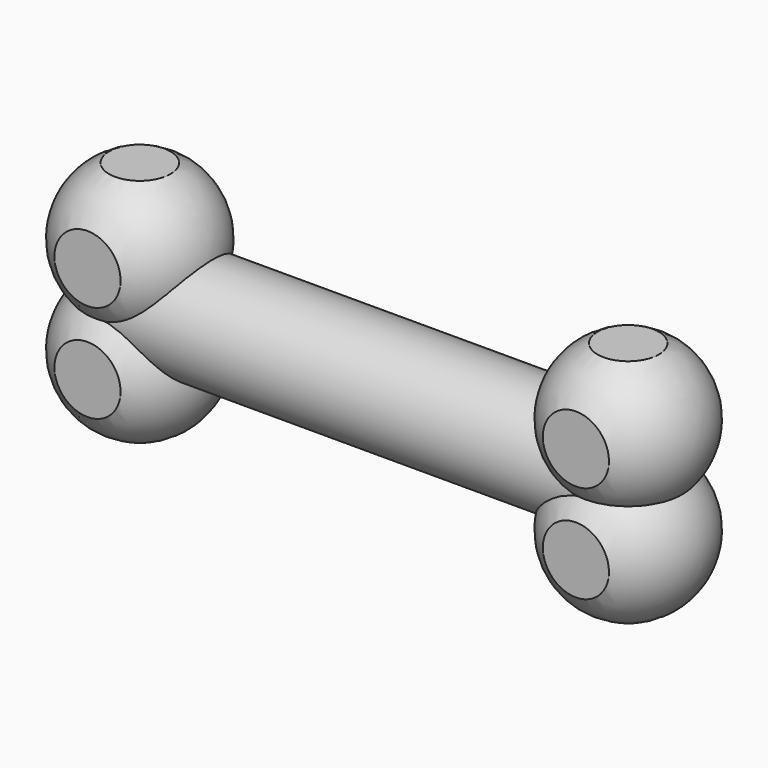
from build123d import *

# Parameters (mm, degrees)
F3_R          = 14
F3_W          = 0.1768313458
F3_H          = 1.6568994889
F3_H_2        = 1.1669505963
F3_W_2        = 0.1419738843
F3_H_3        = 0.9369182155
F3_W_3        = 0.1608024419
F3_H_4        = 1.5067095859
F3_H_5        = 1.0611721842
F3_H_6        = 1.3302870896
F3_W_4        = 0.091749817
F3_H_7        = 0.8596904821
F3_H_8        = 0.6054780796
F3_W_5        = 0.098028363
F3_H_9        = 0.9185200952
F3_W_6        = 0.1414650767
F3_H_10       = 1.3255195911
F3_H_11       = 0.933560477
F3_W_7        = 0.1449230088
F3_H_12       = 0.9563801642
F3_H_13       = 0.6469116443
F3_H_14       = 1.3579202156
F3_W_8        = 0.1300222466
F3_H_15       = 1.2183009349
F3_H_16       = 0.8580466177
F3_W_9        = 0.0875965235
F3_H_17       = 0.820774362
F3_W_10       = 0.0719761238
F3_H_18       = 0.67441212
F3_H_19       = 0.4749869445
F3_H_20       = 0.5780695435
F3_W_11       = 0.0798611688
F3_H_21       = 0.7482945351
F3_H_22       = 0.5270221638
F3_W_12       = 0.0828434925
F3_H_23       = 0.7762387365
F3_H_24       = 0.5467032022
F3_W_13       = 0.1129018001
F3_H_25       = 1.0578833408
F3_H_26       = 0.7450648657
F3_W_14       = 0.059937769
F3_H_27       = 0.5616134313
F3_H_28       = 0.3955430808
F3_W_15       = 0.12155281
F3_H_29       = 1.1389428037
F3_W_16       = 0.0707325383
F3_H_30       = 0.6627597956
F3_W_17       = 0.0796825325
F3_H_31       = 0.7466207235
F3_H_32       = 0.5258433021
F3_H_33       = 0.4667802385
F3_W_18       = 0.0865177565
F3_H_34       = 0.8106663778
F3_H_35       = 0.5709505129
F3_W_19       = 0.1153763794
F3_H_36       = 1.0810700054
F3_H_37       = 0.7613951816
F3_H_38       = 0.8021548638
F4_DEPTH      = 63.5
F5_W          = 54
F5_H          = 80
F5_W_2        = 34
F5_H_2        = 60
F6_DEPTH      = 82.551
F6_DEPTH_BACK = 82.551
F7_TEXT_SIZE  = 10.5435979983
F8_DEPTH      = 25


# Not quite as in the source:
# - Text() gives the source's letters only with a copy of the font that has no kerning and outlines rounded to 1/6400 em; it was checked with that copy


with BuildPart() as f1:
    # F0 (on Front) → F1 (revolve)
    with BuildSketch(Plane.XZ):
        with BuildLine():
            Line((-82.55, 12.7), (-44.45, 12.7))
            ThreePointArc((-44.45, 12.7), (-63.5, 31.75), (-82.55, 12.7))
        make_face()
    revolve(axis=Axis((0, 0, 12.7), (1, 0, 0)))


with BuildPart() as f1b:
    # F0 (on Front) → F1, piece 2 (revolve)
    with BuildSketch(Plane.XZ):
        with BuildLine():
            Line((44.45, 12.7), (82.55, 12.7))
            ThreePointArc((82.55, 12.7), (63.5, 31.75), (44.45, 12.7))
        make_face()
    revolve(axis=Axis((0, 0, 12.7), (1, 0, 0)))


with BuildPart() as f2:
    # F0 (on Front) → F2 (revolve)
    with BuildSketch(Plane.XZ):
        with BuildLine():
            Line((-44.45, -12.7), (-82.55, -12.7))
            ThreePointArc((-82.55, -12.7), (-63.5, -31.75), (-44.45, -12.7))
        make_face()
    revolve(axis=Axis((0, 0, -12.7), (1, 0, 0)))


with BuildPart() as f2b:
    # F0 (on Front) → F2, piece 2 (revolve)
    with BuildSketch(Plane.XZ):
        with BuildLine():
            Line((82.55, -12.7), (44.45, -12.7))
            ThreePointArc((44.45, -12.7), (63.5, -31.75), (82.55, -12.7))
        make_face()
    revolve(axis=Axis((0, 0, -12.7), (1, 0, 0)))


with BuildPart() as f4:
    # F3 (on Right) → F4 (new body, symmetric)
    with BuildSketch(Plane.YZ):
        Circle(F3_R)
        with BuildLine():
            Line((-7.2096864432, -7.5286109932), (-7.3150042572, -7.5286109932))
            Line((-7.3150042572, -7.5286109932), (-7.3431801918, -7.3951172445))
            Line((-7.3431801918, -7.3951172445), (-7.3500190109, -7.3951172445))
            add(Edge.make_bspline(
                [(-7.3500190109, -7.3951172445), (-7.4200485184, -7.4832012344), (-7.4896676968, -7.5145230258)],
                knots=[0, 0, 0, 1, 1, 1], degree=2))
            add(Edge.make_bspline(
                [(-7.4896676968, -7.5145230258), (-7.5592868751, -7.5458448173), (-7.6637840308, -7.5458448173)],
                knots=[0, 0, 0, 1, 1, 1], degree=2))
            add(Edge.make_bspline(
                [(-7.6637840308, -7.5458448173), (-7.8030223875, -7.5458448173), (-7.8820791362, -7.4739004404)],
                knots=[0, 0, 0, 1, 1, 1], degree=2))
            add(Edge.make_bspline(
                [(-7.8820791362, -7.4739004404), (-7.9611358849, -7.4019560636), (-7.9611358849, -7.269556526)],
                knots=[0, 0, 0, 1, 1, 1], degree=2))
            add(Edge.make_bspline(
                [(-7.9611358849, -7.269556526), (-7.9611358849, -6.9858823101), (-7.50731185, -6.9722046719)],
                knots=[0, 0, 0, 1, 1, 1], degree=2))
            Line((-7.50731185, -6.9722046719), (-7.3483776943, -6.9670071694))
            Line((-7.3483776943, -6.9670071694), (-7.3483776943, -6.9087404307))
            add(Edge.make_bspline(
                [(-7.3483776943, -6.9087404307), (-7.3483776943, -6.798498667), (-7.3957023225, -6.7459765364)],
                knots=[0, 0, 0, 1, 1, 1], degree=2))
            add(Edge.make_bspline(
                [(-7.3957023225, -6.7459765364), (-7.4430269506, -6.6934544058), (-7.5475241063, -6.6934544058)],
                knots=[0, 0, 0, 1, 1, 1], degree=2))
            add(Edge.make_bspline(
                [(-7.5475241063, -6.6934544058), (-7.6646046891, -6.6934544058), (-7.8123231815, -6.7651252298)],
                knots=[0, 0, 0, 1, 1, 1], degree=2))
            Line((-7.8123231815, -6.7651252298), (-7.8560916237, -6.6565247827))
            add(Edge.make_bspline(
                [(-7.8560916237, -6.6565247827), (-7.7868827745, -6.619048054), (-7.7044066162, -6.5977109385)],
                knots=[0, 0, 0, 1, 1, 1], degree=2))
            add(Edge.make_bspline(
                [(-7.7044066162, -6.5977109385), (-7.621930458, -6.5763738229), (-7.5387704178, -6.5763738229)],
                knots=[0, 0, 0, 1, 1, 1], degree=2))
            add(Edge.make_bspline(
                [(-7.5387704178, -6.5763738229), (-7.3713561265, -6.5763738229), (-7.2905212848, -6.6506433982)],
                knots=[0, 0, 0, 1, 1, 1], degree=2))
            add(Edge.make_bspline(
                [(-7.2905212848, -6.6506433982), (-7.2096864432, -6.7249129736), (-7.2096864432, -6.8890446318)],
                knots=[0, 0, 0, 1, 1, 1], degree=2))
            Line((-7.2096864432, -6.8890446318), (-7.2096864432, -7.5286109932))
        make_face(mode=Mode.SUBTRACT)
        Polygon((-3.6201022147, -12.2238405542), (-3.8074957411, -12.2238405542), (-4.001362862, -11.7287809289), (-4.6252129472, -11.7287809289), (-4.8166950596, -12.2238405542), (-5, -12.2238405542), (-4.3846678024, -10.6606378284), (-4.2323679727, -10.6606378284), align=None, mode=Mode.SUBTRACT)
        with Locations((-3.3442930153, -11.3953908097)):
            Rectangle(F3_W, F3_H, mode=Mode.SUBTRACT)
        with BuildLine():
            Line((-2.0323679727, -12.2238405542), (-2.1635434412, -12.2238405542))
            Line((-2.1635434412, -12.2238405542), (-2.198637138, -12.0575713889))
            Line((-2.198637138, -12.0575713889), (-2.2071550256, -12.0575713889))
            add(Edge.make_bspline(
                [(-2.2071550256, -12.0575713889), (-2.2943781942, -12.1672817807), (-2.3810902896, -12.2062937058)],
                knots=[0, 0, 0, 1, 1, 1], degree=2))
            add(Edge.make_bspline(
                [(-2.3810902896, -12.2062937058), (-2.467802385, -12.2453056308), (-2.597955707, -12.2453056308)],
                knots=[0, 0, 0, 1, 1, 1], degree=2))
            add(Edge.make_bspline(
                [(-2.597955707, -12.2453056308), (-2.7713798978, -12.2453056308), (-2.869846678, -12.1556974536)],
                knots=[0, 0, 0, 1, 1, 1], degree=2))
            add(Edge.make_bspline(
                [(-2.869846678, -12.1556974536), (-2.9683134583, -12.0660892765), (-2.9683134583, -11.9011829732)],
                knots=[0, 0, 0, 1, 1, 1], degree=2))
            add(Edge.make_bspline(
                [(-2.9683134583, -11.9011829732), (-2.9683134583, -11.5478609971), (-2.4030664395, -11.530825222)],
                knots=[0, 0, 0, 1, 1, 1], degree=2))
            Line((-2.4030664395, -11.530825222), (-2.2051107325, -11.5243516274))
            Line((-2.2051107325, -11.5243516274), (-2.2051107325, -11.4517792254))
            add(Edge.make_bspline(
                [(-2.2051107325, -11.4517792254), (-2.2051107325, -11.3144708778), (-2.2640545145, -11.2490535013)],
                knots=[0, 0, 0, 1, 1, 1], degree=2))
            add(Edge.make_bspline(
                [(-2.2640545145, -11.2490535013), (-2.3229982964, -11.1836361249), (-2.4531516184, -11.1836361249)],
                knots=[0, 0, 0, 1, 1, 1], degree=2))
            add(Edge.make_bspline(
                [(-2.4531516184, -11.1836361249), (-2.5989778535, -11.1836361249), (-2.7829642249, -11.2729035865)],
                knots=[0, 0, 0, 1, 1, 1], degree=2))
            Line((-2.7829642249, -11.2729035865), (-2.8374787053, -11.137639532))
            add(Edge.make_bspline(
                [(-2.8374787053, -11.137639532), (-2.7512776831, -11.0909615082), (-2.6485519591, -11.064385699)],
                knots=[0, 0, 0, 1, 1, 1], degree=2))
            add(Edge.make_bspline(
                [(-2.6485519591, -11.064385699), (-2.5458262351, -11.0378098898), (-2.4422487223, -11.0378098898)],
                knots=[0, 0, 0, 1, 1, 1], degree=2))
            add(Edge.make_bspline(
                [(-2.4422487223, -11.0378098898), (-2.2337308348, -11.0378098898), (-2.1330494037, -11.1303141487)],
                knots=[0, 0, 0, 1, 1, 1], degree=2))
            add(Edge.make_bspline(
                [(-2.1330494037, -11.1303141487), (-2.0323679727, -11.2228184076), (-2.0323679727, -11.4272477092)],
                knots=[0, 0, 0, 1, 1, 1], degree=2))
            Line((-2.0323679727, -11.4272477092), (-2.0323679727, -12.2238405542))
        make_face(mode=Mode.SUBTRACT)
        with Locations((-1.5800681431, -11.640365256)):
            Rectangle(F3_W, F3_H_2, mode=Mode.SUBTRACT)
        with BuildLine():
            Line((-0.1413969336, -12.2238405542), (-0.3182282794, -12.2238405542))
            Line((-0.3182282794, -12.2238405542), (-0.3182282794, -11.4688150005))
            add(Edge.make_bspline(
                [(-0.3182282794, -11.4688150005), (-0.3182282794, -11.3263959204), (-0.3831345826, -11.2560381691)],
                knots=[0, 0, 0, 1, 1, 1], degree=2))
            add(Edge.make_bspline(
                [(-0.3831345826, -11.2560381691), (-0.4480408859, -11.1856804179), (-0.5867120954, -11.1856804179)],
                knots=[0, 0, 0, 1, 1, 1], degree=2))
            add(Edge.make_bspline(
                [(-0.5867120954, -11.1856804179), (-0.7696763203, -11.1856804179), (-0.8548551959, -11.2846582714)],
                knots=[0, 0, 0, 1, 1, 1], degree=2))
            add(Edge.make_bspline(
                [(-0.8548551959, -11.2846582714), (-0.9400340716, -11.3836361249), (-0.9400340716, -11.6115747961)],
                knots=[0, 0, 0, 1, 1, 1], degree=2))
            Line((-0.9400340716, -11.6115747961), (-0.9400340716, -12.2238405542))
            Line((-0.9400340716, -12.2238405542), (-1.1168654174, -12.2238405542))
            Line((-1.1168654174, -12.2238405542), (-1.1168654174, -11.0568899579))
            Line((-1.1168654174, -11.0568899579), (-0.9730834753, -11.0568899579))
            Line((-0.9730834753, -11.0568899579), (-0.9444633731, -11.2166855286))
            Line((-0.9444633731, -11.2166855286), (-0.9359454855, -11.2166855286))
            add(Edge.make_bspline(
                [(-0.9359454855, -11.2166855286), (-0.8814310051, -11.1304845065), (-0.7834752981, -11.0829546938)],
                knots=[0, 0, 0, 1, 1, 1], degree=2))
            add(Edge.make_bspline(
                [(-0.7834752981, -11.0829546938), (-0.6855195911, -11.0354248812), (-0.5652470187, -11.0354248812)],
                knots=[0, 0, 0, 1, 1, 1], degree=2))
            add(Edge.make_bspline(
                [(-0.5652470187, -11.0354248812), (-0.3543441227, -11.0354248812), (-0.2478705281, -11.1371284588)],
                knots=[0, 0, 0, 1, 1, 1], degree=2))
            add(Edge.make_bspline(
                [(-0.2478705281, -11.1371284588), (-0.1413969336, -11.2388320363), (-0.1413969336, -11.4626821214)],
                knots=[0, 0, 0, 1, 1, 1], degree=2))
            Line((-0.1413969336, -11.4626821214), (-0.1413969336, -12.2238405542))
        make_face(mode=Mode.SUBTRACT)
        with BuildLine():
            add(Edge.make_bspline(
                [(-1.6536626917, -10.8296327177), (-1.6834752981, -10.8003311845), (-1.6834752981, -10.7407059715)],
                knots=[0, 0, 0, 1, 1, 1], degree=2))
            add(Edge.make_bspline(
                [(-1.6834752981, -10.7407059715), (-1.6834752981, -10.6800586121), (-1.6536626917, -10.6517792254)],
                knots=[0, 0, 0, 1, 1, 1], degree=2))
            add(Edge.make_bspline(
                [(-1.6536626917, -10.6517792254), (-1.6238500852, -10.6234998387), (-1.5788756388, -10.6234998387)],
                knots=[0, 0, 0, 1, 1, 1], degree=2))
            add(Edge.make_bspline(
                [(-1.5788756388, -10.6234998387), (-1.536286201, -10.6234998387), (-1.505451448, -10.6522902986)],
                knots=[0, 0, 0, 1, 1, 1], degree=2))
            add(Edge.make_bspline(
                [(-1.505451448, -10.6522902986), (-1.4746166951, -10.6810807586), (-1.4746166951, -10.7407059715)],
                knots=[0, 0, 0, 1, 1, 1], degree=2))
            add(Edge.make_bspline(
                [(-1.4746166951, -10.7407059715), (-1.4746166951, -10.8003311845), (-1.505451448, -10.8296327177)],
                knots=[0, 0, 0, 1, 1, 1], degree=2))
            add(Edge.make_bspline(
                [(-1.505451448, -10.8296327177), (-1.536286201, -10.8589342509), (-1.5788756388, -10.8589342509)],
                knots=[0, 0, 0, 1, 1, 1], degree=2))
            add(Edge.make_bspline(
                [(-1.5788756388, -10.8589342509), (-1.6238500852, -10.8589342509), (-1.6536626917, -10.8296327177)],
                knots=[0, 0, 0, 1, 1, 1], degree=2))
        make_face(mode=Mode.SUBTRACT)
        with Locations((-6.8465451494, -7.0601518854)):
            Rectangle(F3_W_2, F3_H_3, mode=Mode.SUBTRACT)
        with BuildLine():
            Line((-5.6914686049, -7.5286109932), (-5.8334424892, -7.5286109932))
            Line((-5.8334424892, -7.5286109932), (-5.8334424892, -6.9224180689))
            add(Edge.make_bspline(
                [(-5.8334424892, -6.9224180689), (-5.8334424892, -6.8080730137), (-5.8855542907, -6.751584368)],
                knots=[0, 0, 0, 1, 1, 1], degree=2))
            add(Edge.make_bspline(
                [(-5.8855542907, -6.751584368), (-5.9376660922, -6.6950957223), (-6.049002067, -6.6950957223)],
                knots=[0, 0, 0, 1, 1, 1], degree=2))
            add(Edge.make_bspline(
                [(-6.049002067, -6.6950957223), (-6.1958999011, -6.6950957223), (-6.264288092, -6.7745628002)],
                knots=[0, 0, 0, 1, 1, 1], degree=2))
            add(Edge.make_bspline(
                [(-6.264288092, -6.7745628002), (-6.3326762829, -6.854029878), (-6.3326762829, -7.0370366769)],
                knots=[0, 0, 0, 1, 1, 1], degree=2))
            Line((-6.3326762829, -7.0370366769), (-6.3326762829, -7.5286109932))
            Line((-6.3326762829, -7.5286109932), (-6.4746501672, -7.5286109932))
            Line((-6.4746501672, -7.5286109932), (-6.4746501672, -6.5916927777))
            Line((-6.4746501672, -6.5916927777), (-6.359210901, -6.5916927777))
            Line((-6.359210901, -6.5916927777), (-6.3362324688, -6.7199890238))
            Line((-6.3362324688, -6.7199890238), (-6.3293936497, -6.7199890238))
            add(Edge.make_bspline(
                [(-6.3293936497, -6.7199890238), (-6.2856252076, -6.6507801746), (-6.206978788, -6.6126195641)],
                knots=[0, 0, 0, 1, 1, 1], degree=2))
            add(Edge.make_bspline(
                [(-6.206978788, -6.6126195641), (-6.1283323685, -6.5744589536), (-6.0317682429, -6.5744589536)],
                knots=[0, 0, 0, 1, 1, 1], degree=2))
            add(Edge.make_bspline(
                [(-6.0317682429, -6.5744589536), (-5.8624390822, -6.5744589536), (-5.7769538436, -6.6561144535)],
                knots=[0, 0, 0, 1, 1, 1], degree=2))
            add(Edge.make_bspline(
                [(-5.7769538436, -6.6561144535), (-5.6914686049, -6.7377699535), (-5.6914686049, -6.9174941192)],
                knots=[0, 0, 0, 1, 1, 1], degree=2))
            Line((-5.6914686049, -6.9174941192), (-5.6914686049, -7.5286109932))
        make_face(mode=Mode.SUBTRACT)
        Polygon((-2.4357838847, -10.1848877966), (-2.6061910968, -10.1848877966), (-2.7824851034, -9.7347029255), (-3.3497862039, -9.7347029255), (-3.5239113915, -10.1848877966), (-3.690600628, -10.1848877966), (-3.1310453099, -8.7633818168), (-2.9925507212, -8.7633818168), align=None, mode=Mode.SUBTRACT)
        with Locations((-2.1849754517, -9.4315330037)):
            Rectangle(F3_W_3, F3_H_4, mode=Mode.SUBTRACT)
        with BuildLine():
            Line((-0.9919700517, -10.1848877966), (-1.1112551001, -10.1848877966))
            Line((-1.1112551001, -10.1848877966), (-1.1431677235, -10.0336901249))
            Line((-1.1431677235, -10.0336901249), (-1.1509135058, -10.0336901249))
            add(Edge.make_bspline(
                [(-1.1509135058, -10.0336901249), (-1.2302303173, -10.1334558017), (-1.3090823817, -10.168931485)],
                knots=[0, 0, 0, 1, 1, 1], degree=2))
            add(Edge.make_bspline(
                [(-1.3090823817, -10.168931485), (-1.3879344462, -10.2044071682), (-1.5062900008, -10.2044071682)],
                knots=[0, 0, 0, 1, 1, 1], degree=2))
            add(Edge.make_bspline(
                [(-1.5062900008, -10.2044071682), (-1.6639941298, -10.2044071682), (-1.7535353739, -10.1229215377)],
                knots=[0, 0, 0, 1, 1, 1], degree=2))
            add(Edge.make_bspline(
                [(-1.7535353739, -10.1229215377), (-1.8430766181, -10.0414359072), (-1.8430766181, -9.8914775606)],
                knots=[0, 0, 0, 1, 1, 1], degree=2))
            add(Edge.make_bspline(
                [(-1.8430766181, -9.8914775606), (-1.8430766181, -9.5701825081), (-1.3290665002, -9.5546909433)],
                knots=[0, 0, 0, 1, 1, 1], degree=2))
            Line((-1.3290665002, -9.5546909433), (-1.1490545181, -9.5488041487))
            Line((-1.1490545181, -9.5488041487), (-1.1490545181, -9.482810083))
            add(Edge.make_bspline(
                [(-1.1490545181, -9.482810083), (-1.1490545181, -9.3579480712), (-1.202655332, -9.2984604627)],
                knots=[0, 0, 0, 1, 1, 1], degree=2))
            add(Edge.make_bspline(
                [(-1.202655332, -9.2984604627), (-1.256256146, -9.2389728541), (-1.3746117006, -9.2389728541)],
                knots=[0, 0, 0, 1, 1, 1], degree=2))
            add(Edge.make_bspline(
                [(-1.3746117006, -9.2389728541), (-1.5072194947, -9.2389728541), (-1.6745283938, -9.3201486533)],
                knots=[0, 0, 0, 1, 1, 1], degree=2))
            Line((-1.6745283938, -9.3201486533), (-1.7241014009, -9.1971456293))
            add(Edge.make_bspline(
                [(-1.7241014009, -9.1971456293), (-1.6457140834, -9.1546987419), (-1.552299948, -9.130531901)],
                knots=[0, 0, 0, 1, 1, 1], degree=2))
            add(Edge.make_bspline(
                [(-1.552299948, -9.130531901), (-1.4588858127, -9.10636506), (-1.3646970991, -9.10636506)],
                knots=[0, 0, 0, 1, 1, 1], degree=2))
            add(Edge.make_bspline(
                [(-1.3646970991, -9.10636506), (-1.1750803468, -9.10636506), (-1.0835251992, -9.1904842565)],
                knots=[0, 0, 0, 1, 1, 1], degree=2))
            add(Edge.make_bspline(
                [(-1.0835251992, -9.1904842565), (-0.9919700517, -9.274603453), (-0.9919700517, -9.4605022298)],
                knots=[0, 0, 0, 1, 1, 1], degree=2))
            Line((-0.9919700517, -9.4605022298), (-0.9919700517, -10.1848877966))
        make_face(mode=Mode.SUBTRACT)
        with Locations((-0.580669008, -9.6543017046)):
            Rectangle(F3_W_3, F3_H_5, mode=Mode.SUBTRACT)
        with BuildLine():
            add(Edge.make_bspline(
                [(-0.6475925677, -8.917058139), (-0.674702806, -8.8904126476), (-0.674702806, -8.8361921711)],
                knots=[0, 0, 0, 1, 1, 1], degree=2))
            add(Edge.make_bspline(
                [(-0.674702806, -8.8361921711), (-0.674702806, -8.7810422006), (-0.6475925677, -8.7553262031)],
                knots=[0, 0, 0, 1, 1, 1], degree=2))
            add(Edge.make_bspline(
                [(-0.6475925677, -8.7553262031), (-0.6204823294, -8.7296102057), (-0.5795845985, -8.7296102057)],
                knots=[0, 0, 0, 1, 1, 1], degree=2))
            add(Edge.make_bspline(
                [(-0.5795845985, -8.7296102057), (-0.5408556867, -8.7296102057), (-0.5128159545, -8.7557909501)],
                knots=[0, 0, 0, 1, 1, 1], degree=2))
            add(Edge.make_bspline(
                [(-0.5128159545, -8.7557909501), (-0.4847762223, -8.7819716945), (-0.4847762223, -8.8361921711)],
                knots=[0, 0, 0, 1, 1, 1], degree=2))
            add(Edge.make_bspline(
                [(-0.4847762223, -8.8361921711), (-0.4847762223, -8.8904126476), (-0.5128159545, -8.917058139)],
                knots=[0, 0, 0, 1, 1, 1], degree=2))
            add(Edge.make_bspline(
                [(-0.5128159545, -8.917058139), (-0.5408556867, -8.9437036303), (-0.5795845985, -8.9437036303)],
                knots=[0, 0, 0, 1, 1, 1], degree=2))
            add(Edge.make_bspline(
                [(-0.5795845985, -8.9437036303), (-0.6204823294, -8.9437036303), (-0.6475925677, -8.917058139)],
                knots=[0, 0, 0, 1, 1, 1], degree=2))
        make_face(mode=Mode.SUBTRACT)
        Polygon((-8.4844423218, -7.5286109932), (-8.6348963418, -7.5286109932), (-8.7905478643, -7.1311388276), (-9.2914229746, -7.1311388276), (-9.4451596277, -7.5286109932), (-9.5923310146, -7.5286109932), (-9.0982947234, -6.2735509135), (-8.9760166381, -6.2735509135), align=None, mode=Mode.SUBTRACT)
        with Locations((-8.2630013596, -6.8634674484)):
            Rectangle(F3_W_2, F3_H_6, mode=Mode.SUBTRACT)
        Polygon((-11.1035979571, -3.3536257688), (-11.2008280137, -3.3536257688), (-11.3014169268, -3.0967616375), (-11.6251046242, -3.0967616375), (-11.7244560639, -3.3536257688), (-11.8195647374, -3.3536257688), (-11.500296588, -2.542550315), (-11.4212750692, -2.542550315), align=None, mode=Mode.SUBTRACT)
        with Locations((-10.960492992, -2.9237805278)):
            Rectangle(F3_W_4, F3_H_7, mode=Mode.SUBTRACT)
        with BuildLine():
            Line((-10.279794205, -3.3536257688), (-10.3478552446, -3.3536257688))
            Line((-10.3478552446, -3.3536257688), (-10.3660637825, -3.2673561913))
            Line((-10.3660637825, -3.2673561913), (-10.3704833305, -3.2673561913))
            add(Edge.make_bspline(
                [(-10.3704833305, -3.2673561913), (-10.4157395023, -3.3242799699), (-10.4607305012, -3.3445214999)],
                knots=[0, 0, 0, 1, 1, 1], degree=2))
            add(Edge.make_bspline(
                [(-10.4607305012, -3.3445214999), (-10.5057215001, -3.3647630298), (-10.573252194, -3.3647630298)],
                knots=[0, 0, 0, 1, 1, 1], degree=2))
            add(Edge.make_bspline(
                [(-10.573252194, -3.3647630298), (-10.6632341918, -3.3647630298), (-10.714324167, -3.3182693846)],
                knots=[0, 0, 0, 1, 1, 1], degree=2))
            add(Edge.make_bspline(
                [(-10.714324167, -3.3182693846), (-10.7654141421, -3.2717757393), (-10.7654141421, -3.1862132896)],
                knots=[0, 0, 0, 1, 1, 1], degree=2))
            add(Edge.make_bspline(
                [(-10.7654141421, -3.1862132896), (-10.7654141421, -3.0028904374), (-10.4721329351, -2.9940513414)],
                knots=[0, 0, 0, 1, 1, 1], degree=2))
            Line((-10.4721329351, -2.9940513414), (-10.369422639, -2.9906924849))
            Line((-10.369422639, -2.9906924849), (-10.369422639, -2.9530379357))
            add(Edge.make_bspline(
                [(-10.369422639, -2.9530379357), (-10.369422639, -2.8817948215), (-10.4000059113, -2.8478526927)],
                knots=[0, 0, 0, 1, 1, 1], degree=2))
            add(Edge.make_bspline(
                [(-10.4000059113, -2.8478526927), (-10.4305891837, -2.8139105638), (-10.4981198775, -2.8139105638)],
                knots=[0, 0, 0, 1, 1, 1], degree=2))
            add(Edge.make_bspline(
                [(-10.4981198775, -2.8139105638), (-10.5737825397, -2.8139105638), (-10.6692447771, -2.8602274271)],
                knots=[0, 0, 0, 1, 1, 1], degree=2))
            Line((-10.6692447771, -2.8602274271), (-10.6975298845, -2.7900450045))
            add(Edge.make_bspline(
                [(-10.6975298845, -2.7900450045), (-10.6528040584, -2.7658258813), (-10.5995043092, -2.7520368915)],
                knots=[0, 0, 0, 1, 1, 1], degree=2))
            add(Edge.make_bspline(
                [(-10.5995043092, -2.7520368915), (-10.54620456, -2.7382479016), (-10.492462856, -2.7382479016)],
                knots=[0, 0, 0, 1, 1, 1], degree=2))
            add(Edge.make_bspline(
                [(-10.492462856, -2.7382479016), (-10.3842723204, -2.7382479016), (-10.3320332627, -2.7862441932)],
                knots=[0, 0, 0, 1, 1, 1], degree=2))
            add(Edge.make_bspline(
                [(-10.3320332627, -2.7862441932), (-10.279794205, -2.8342404847), (-10.279794205, -2.9403096374)],
                knots=[0, 0, 0, 1, 1, 1], degree=2))
            Line((-10.279794205, -2.9403096374), (-10.279794205, -3.3536257688))
        make_face(mode=Mode.SUBTRACT)
        with Locations((-10.0451162048, -3.050886729)):
            Rectangle(F3_W_4, F3_H_8, mode=Mode.SUBTRACT)
        with BuildLine():
            Line((-9.2986545432, -3.3536257688), (-9.3904043602, -3.3536257688))
            Line((-9.3904043602, -3.3536257688), (-9.3904043602, -2.9618770317))
            add(Edge.make_bspline(
                [(-9.3904043602, -2.9618770317), (-9.3904043602, -2.8879821887), (-9.4240813162, -2.851476722)],
                knots=[0, 0, 0, 1, 1, 1], degree=2))
            add(Edge.make_bspline(
                [(-9.4240813162, -2.851476722), (-9.4577582721, -2.8149712553), (-9.529708514, -2.8149712553)],
                knots=[0, 0, 0, 1, 1, 1], degree=2))
            add(Edge.make_bspline(
                [(-9.529708514, -2.8149712553), (-9.6246404056, -2.8149712553), (-9.6688358859, -2.8663264034)],
                knots=[0, 0, 0, 1, 1, 1], degree=2))
            add(Edge.make_bspline(
                [(-9.6688358859, -2.8663264034), (-9.7130313661, -2.9176815515), (-9.7130313661, -3.0359486567)],
                knots=[0, 0, 0, 1, 1, 1], degree=2))
            Line((-9.7130313661, -3.0359486567), (-9.7130313661, -3.3536257688))
            Line((-9.7130313661, -3.3536257688), (-9.8047811831, -3.3536257688))
            Line((-9.8047811831, -3.3536257688), (-9.8047811831, -2.7481476892))
            Line((-9.8047811831, -2.7481476892), (-9.7301792125, -2.7481476892))
            Line((-9.7301792125, -2.7481476892), (-9.7153295311, -2.8310584102))
            Line((-9.7153295311, -2.8310584102), (-9.7109099831, -2.8310584102))
            add(Edge.make_bspline(
                [(-9.7109099831, -2.8310584102), (-9.6826248757, -2.7863325841), (-9.6318000734, -2.7616715062)],
                knots=[0, 0, 0, 1, 1, 1], degree=2))
            add(Edge.make_bspline(
                [(-9.6318000734, -2.7616715062), (-9.5809752711, -2.7370104282), (-9.518571253, -2.7370104282)],
                knots=[0, 0, 0, 1, 1, 1], degree=2))
            add(Edge.make_bspline(
                [(-9.518571253, -2.7370104282), (-9.4091432438, -2.7370104282), (-9.3538988935, -2.7897798316)],
                knots=[0, 0, 0, 1, 1, 1], degree=2))
            add(Edge.make_bspline(
                [(-9.3538988935, -2.7897798316), (-9.2986545432, -2.842549235), (-9.2986545432, -2.9586949572)],
                knots=[0, 0, 0, 1, 1, 1], degree=2))
            Line((-9.2986545432, -2.9586949572), (-9.2986545432, -3.3536257688))
        make_face(mode=Mode.SUBTRACT)
        with BuildLine():
            add(Edge.make_bspline(
                [(-10.0833010998, -2.6302341478), (-10.0987695179, -2.6150309026), (-10.0987695179, -2.5840940665)],
                knots=[0, 0, 0, 1, 1, 1], degree=2))
            add(Edge.make_bspline(
                [(-10.0987695179, -2.5840940665), (-10.0987695179, -2.5526268845), (-10.0833010998, -2.5379539851)],
                knots=[0, 0, 0, 1, 1, 1], degree=2))
            add(Edge.make_bspline(
                [(-10.0833010998, -2.5379539851), (-10.0678326817, -2.5232810856), (-10.0444974681, -2.5232810856)],
                knots=[0, 0, 0, 1, 1, 1], degree=2))
            add(Edge.make_bspline(
                [(-10.0444974681, -2.5232810856), (-10.022399728, -2.5232810856), (-10.0064009641, -2.5382191579)],
                knots=[0, 0, 0, 1, 1, 1], degree=2))
            add(Edge.make_bspline(
                [(-10.0064009641, -2.5382191579), (-9.9904022002, -2.5531572303), (-9.9904022002, -2.5840940665)],
                knots=[0, 0, 0, 1, 1, 1], degree=2))
            add(Edge.make_bspline(
                [(-9.9904022002, -2.5840940665), (-9.9904022002, -2.6150309026), (-10.0064009641, -2.6302341478)],
                knots=[0, 0, 0, 1, 1, 1], degree=2))
            add(Edge.make_bspline(
                [(-10.0064009641, -2.6302341478), (-10.022399728, -2.6454373931), (-10.0444974681, -2.6454373931)],
                knots=[0, 0, 0, 1, 1, 1], degree=2))
            add(Edge.make_bspline(
                [(-10.0444974681, -2.6454373931), (-10.0678326817, -2.6454373931), (-10.0833010998, -2.6302341478)],
                knots=[0, 0, 0, 1, 1, 1], degree=2))
        make_face(mode=Mode.SUBTRACT)
        with BuildLine():
            add(Edge.make_bspline(
                [(-6.9056325464, -6.4092330843), (-6.9295684132, -6.3857075466), (-6.9295684132, -6.337835813)],
                knots=[0, 0, 0, 1, 1, 1], degree=2))
            add(Edge.make_bspline(
                [(-6.9295684132, -6.337835813), (-6.9295684132, -6.2891434211), (-6.9056325464, -6.2664385417)],
                knots=[0, 0, 0, 1, 1, 1], degree=2))
            add(Edge.make_bspline(
                [(-6.9056325464, -6.2664385417), (-6.8816966796, -6.2437336623), (-6.8455877148, -6.2437336623)],
                knots=[0, 0, 0, 1, 1, 1], degree=2))
            add(Edge.make_bspline(
                [(-6.8455877148, -6.2437336623), (-6.8113936193, -6.2437336623), (-6.7866370942, -6.2668488708)],
                knots=[0, 0, 0, 1, 1, 1], degree=2))
            add(Edge.make_bspline(
                [(-6.7866370942, -6.2668488708), (-6.7618805691, -6.2899640794), (-6.7618805691, -6.337835813)],
                knots=[0, 0, 0, 1, 1, 1], degree=2))
            add(Edge.make_bspline(
                [(-6.7618805691, -6.337835813), (-6.7618805691, -6.3857075466), (-6.7866370942, -6.4092330843)],
                knots=[0, 0, 0, 1, 1, 1], degree=2))
            add(Edge.make_bspline(
                [(-6.7866370942, -6.4092330843), (-6.8113936193, -6.432758622), (-6.8455877148, -6.432758622)],
                knots=[0, 0, 0, 1, 1, 1], degree=2))
            add(Edge.make_bspline(
                [(-6.8455877148, -6.432758622), (-6.8816966796, -6.432758622), (-6.9056325464, -6.4092330843)],
                knots=[0, 0, 0, 1, 1, 1], degree=2))
        make_face(mode=Mode.SUBTRACT)
        Polygon((-0.5641851112, -6.7550642416), (-0.6680687329, -6.7550642416), (-0.7755410616, -6.480622601), (-1.1213790822, -6.480622601), (-1.2275292556, -6.7550642416), (-1.3291463256, -6.7550642416), (-0.9880302878, -5.8884859573), (-0.9036012352, -5.8884859573), align=None, mode=Mode.SUBTRACT)
        with Locations((-0.411287308, -6.295804194)):
            Rectangle(F3_W_5, F3_H_9, mode=Mode.SUBTRACT)
        Polygon((2.4135733694, -11.5387545569), (2.2636585482, -11.5387545569), (2.1085648515, -11.1427068567), (1.6094847833, -11.1427068567), (1.4562990934, -11.5387545569), (1.3096551411, -11.5387545569), (1.8019208992, -10.2881923763), (1.9237607629, -10.2881923763), align=None, mode=Mode.SUBTRACT)
        with BuildLine():
            Line((3.6837607629, -11.5387545569), (3.5788203881, -11.5387545569))
            Line((3.5788203881, -11.5387545569), (3.5507454307, -11.4057392247))
            Line((3.5507454307, -11.4057392247), (3.5439311206, -11.4057392247))
            add(Edge.make_bspline(
                [(3.5439311206, -11.4057392247), (3.4741525857, -11.4935075381), (3.4047829094, -11.5247170781)],
                knots=[0, 0, 0, 1, 1, 1], degree=2))
            add(Edge.make_bspline(
                [(3.4047829094, -11.5247170781), (3.3354132331, -11.5559266182), (3.2312905755, -11.5559266182)],
                knots=[0, 0, 0, 1, 1, 1], degree=2))
            add(Edge.make_bspline(
                [(3.2312905755, -11.5559266182), (3.0925512229, -11.5559266182), (3.0137777987, -11.4842400764)],
                knots=[0, 0, 0, 1, 1, 1], degree=2))
            add(Edge.make_bspline(
                [(3.0137777987, -11.4842400764), (2.9350043745, -11.4125535347), (2.9350043745, -11.2806284921)],
                knots=[0, 0, 0, 1, 1, 1], degree=2))
            add(Edge.make_bspline(
                [(2.9350043745, -11.2806284921), (2.9350043745, -10.9979709112), (3.3872019895, -10.9843422911)],
                knots=[0, 0, 0, 1, 1, 1], degree=2))
            Line((3.3872019895, -10.9843422911), (3.5455665551, -10.9791634155))
            Line((3.5455665551, -10.9791634155), (3.5455665551, -10.9211054938))
            add(Edge.make_bspline(
                [(3.5455665551, -10.9211054938), (3.5455665551, -10.8112588158), (3.4984115295, -10.7589249146)],
                knots=[0, 0, 0, 1, 1, 1], degree=2))
            add(Edge.make_bspline(
                [(3.4984115295, -10.7589249146), (3.4512565039, -10.7065910134), (3.3471338464, -10.7065910134)],
                knots=[0, 0, 0, 1, 1, 1], degree=2))
            add(Edge.make_bspline(
                [(3.3471338464, -10.7065910134), (3.2304728583, -10.7065910134), (3.0832837612, -10.7780049827)],
                knots=[0, 0, 0, 1, 1, 1], degree=2))
            Line((3.0832837612, -10.7780049827), (3.0396721769, -10.6697937391))
            add(Edge.make_bspline(
                [(3.0396721769, -10.6697937391), (3.1086329946, -10.6324513201), (3.1908135738, -10.6111906727)],
                knots=[0, 0, 0, 1, 1, 1], degree=2))
            add(Edge.make_bspline(
                [(3.1908135738, -10.6111906727), (3.272994153, -10.5899300253), (3.3558561632, -10.5899300253)],
                knots=[0, 0, 0, 1, 1, 1], degree=2))
            add(Edge.make_bspline(
                [(3.3558561632, -10.5899300253), (3.5226704733, -10.5899300253), (3.6032156181, -10.6639334325)],
                knots=[0, 0, 0, 1, 1, 1], degree=2))
            add(Edge.make_bspline(
                [(3.6032156181, -10.6639334325), (3.6837607629, -10.7379368396), (3.6837607629, -10.9014802809)],
                knots=[0, 0, 0, 1, 1, 1], degree=2))
            Line((3.6837607629, -10.9014802809), (3.6837607629, -11.5387545569))
        make_face(mode=Mode.SUBTRACT)
        with Locations((2.6342207288, -10.8759947613)):
            Rectangle(F3_W_6, F3_H_10, mode=Mode.SUBTRACT)
        with Locations((4.0456006266, -11.0719743184)):
            Rectangle(F3_W_6, F3_H_11, mode=Mode.SUBTRACT)
        with BuildLine():
            Line((5.1965375942, -11.5387545569), (5.0550725176, -11.5387545569))
            Line((5.0550725176, -11.5387545569), (5.0550725176, -10.9347341139))
            add(Edge.make_bspline(
                [(5.0550725176, -10.9347341139), (5.0550725176, -10.8207988499), (5.003147475, -10.7645126488)],
                knots=[0, 0, 0, 1, 1, 1], degree=2))
            add(Edge.make_bspline(
                [(5.003147475, -10.7645126488), (4.9512224324, -10.7082264478), (4.8402854648, -10.7082264478)],
                knots=[0, 0, 0, 1, 1, 1], degree=2))
            add(Edge.make_bspline(
                [(4.8402854648, -10.7082264478), (4.6939140849, -10.7082264478), (4.6257709844, -10.7874087306)],
                knots=[0, 0, 0, 1, 1, 1], degree=2))
            add(Edge.make_bspline(
                [(4.6257709844, -10.7874087306), (4.5576278838, -10.8665910134), (4.5576278838, -11.0489419504)],
                knots=[0, 0, 0, 1, 1, 1], degree=2))
            Line((4.5576278838, -11.0489419504), (4.5576278838, -11.5387545569))
            Line((4.5576278838, -11.5387545569), (4.4161628072, -11.5387545569))
            Line((4.4161628072, -11.5387545569), (4.4161628072, -10.6051940799))
            Line((4.4161628072, -10.6051940799), (4.5311883608, -10.6051940799))
            Line((4.5311883608, -10.6051940799), (4.5540844426, -10.7330305364))
            Line((4.5540844426, -10.7330305364), (4.5608987527, -10.7330305364))
            add(Edge.make_bspline(
                [(4.5608987527, -10.7330305364), (4.604510337, -10.6640697187), (4.6828749026, -10.6260458686)],
                knots=[0, 0, 0, 1, 1, 1], degree=2))
            add(Edge.make_bspline(
                [(4.6828749026, -10.6260458686), (4.7612394682, -10.5880220185), (4.8574575261, -10.5880220185)],
                knots=[0, 0, 0, 1, 1, 1], degree=2))
            add(Edge.make_bspline(
                [(4.8574575261, -10.5880220185), (5.026179843, -10.5880220185), (5.1113587186, -10.6693848805)],
                knots=[0, 0, 0, 1, 1, 1], degree=2))
            add(Edge.make_bspline(
                [(5.1113587186, -10.6693848805), (5.1965375942, -10.7507477425), (5.1965375942, -10.9298278107)],
                knots=[0, 0, 0, 1, 1, 1], degree=2))
            Line((5.1965375942, -10.9298278107), (5.1965375942, -11.5387545569))
        make_face(mode=Mode.SUBTRACT)
        with BuildLine():
            Line((0.7275936336, -10.1848877966), (0.5667911917, -10.1848877966))
            Line((0.5667911917, -10.1848877966), (0.5667911917, -9.4983016477))
            add(Edge.make_bspline(
                [(0.5667911917, -9.4983016477), (0.5667911917, -9.3687921665), (0.5077683301, -9.3048120042)],
                knots=[0, 0, 0, 1, 1, 1], degree=2))
            add(Edge.make_bspline(
                [(0.5077683301, -9.3048120042), (0.4487454684, -9.2408318419), (0.3226441315, -9.2408318419)],
                knots=[0, 0, 0, 1, 1, 1], degree=2))
            add(Edge.make_bspline(
                [(0.3226441315, -9.2408318419), (0.1562647263, -9.2408318419), (0.0788069026, -9.330837833)],
                knots=[0, 0, 0, 1, 1, 1], degree=2))
            add(Edge.make_bspline(
                [(0.0788069026, -9.330837833), (0.001349079, -9.420843824), (0.001349079, -9.6281209602)],
                knots=[0, 0, 0, 1, 1, 1], degree=2))
            Line((0.001349079, -9.6281209602), (0.001349079, -10.1848877966))
            Line((0.001349079, -10.1848877966), (-0.159453363, -10.1848877966))
            Line((-0.159453363, -10.1848877966), (-0.159453363, -9.1237156125))
            Line((-0.159453363, -9.1237156125), (-0.0287045566, -9.1237156125))
            Line((-0.0287045566, -9.1237156125), (-0.0026787279, -9.2690264897))
            Line((-0.0026787279, -9.2690264897), (0.0050670545, -9.2690264897))
            add(Edge.make_bspline(
                [(0.0050670545, -9.2690264897), (0.0546400616, -9.1906391721), (0.1437165588, -9.1474177065)],
                knots=[0, 0, 0, 1, 1, 1], degree=2))
            add(Edge.make_bspline(
                [(0.1437165588, -9.1474177065), (0.2327930561, -9.1041962409), (0.3421635031, -9.1041962409)],
                knots=[0, 0, 0, 1, 1, 1], degree=2))
            add(Edge.make_bspline(
                [(0.3421635031, -9.1041962409), (0.5339490745, -9.1041962409), (0.630771354, -9.1966808824)],
                knots=[0, 0, 0, 1, 1, 1], degree=2))
            add(Edge.make_bspline(
                [(0.630771354, -9.1966808824), (0.7275936336, -9.2891655238), (0.7275936336, -9.4927246844)],
                knots=[0, 0, 0, 1, 1, 1], degree=2))
            Line((0.7275936336, -9.4927246844), (0.7275936336, -10.1848877966))
        make_face(mode=Mode.SUBTRACT)
        with BuildLine():
            add(Edge.make_bspline(
                [(3.9867249878, -10.4233882877), (3.9628749026, -10.3999470611), (3.9628749026, -10.3522468908)],
                knots=[0, 0, 0, 1, 1, 1], degree=2))
            add(Edge.make_bspline(
                [(3.9628749026, -10.3522468908), (3.9628749026, -10.3037290032), (3.9867249878, -10.2811054938)],
                knots=[0, 0, 0, 1, 1, 1], degree=2))
            add(Edge.make_bspline(
                [(3.9867249878, -10.2811054938), (4.0105750729, -10.2584819845), (4.04655463, -10.2584819845)],
                knots=[0, 0, 0, 1, 1, 1], degree=2))
            add(Edge.make_bspline(
                [(4.04655463, -10.2584819845), (4.0806261803, -10.2584819845), (4.1052939827, -10.2815143524)],
                knots=[0, 0, 0, 1, 1, 1], degree=2))
            add(Edge.make_bspline(
                [(4.1052939827, -10.2815143524), (4.129961785, -10.3045467204), (4.129961785, -10.3522468908)],
                knots=[0, 0, 0, 1, 1, 1], degree=2))
            add(Edge.make_bspline(
                [(4.129961785, -10.3522468908), (4.129961785, -10.3999470611), (4.1052939827, -10.4233882877)],
                knots=[0, 0, 0, 1, 1, 1], degree=2))
            add(Edge.make_bspline(
                [(4.1052939827, -10.4233882877), (4.0806261803, -10.4468295143), (4.04655463, -10.4468295143)],
                knots=[0, 0, 0, 1, 1, 1], degree=2))
            add(Edge.make_bspline(
                [(4.04655463, -10.4468295143), (4.0105750729, -10.4468295143), (3.9867249878, -10.4233882877)],
                knots=[0, 0, 0, 1, 1, 1], degree=2))
        make_face(mode=Mode.SUBTRACT)
        with BuildLine():
            Line((7.9922516339, -7.5771021657), (7.8847461264, -7.5771021657))
            Line((7.8847461264, -7.5771021657), (7.8559849127, -7.4408354445))
            Line((7.8559849127, -7.4408354445), (7.8490040356, -7.4408354445))
            add(Edge.make_bspline(
                [(7.8490040356, -7.4408354445), (7.7775198539, -7.5307491417), (7.706454525, -7.5627215588)],
                knots=[0, 0, 0, 1, 1, 1], degree=2))
            add(Edge.make_bspline(
                [(7.706454525, -7.5627215588), (7.635389196, -7.594693976), (7.5287213937, -7.594693976)],
                knots=[0, 0, 0, 1, 1, 1], degree=2))
            add(Edge.make_bspline(
                [(7.5287213937, -7.594693976), (7.3865907357, -7.594693976), (7.3058917963, -7.5212551488)],
                knots=[0, 0, 0, 1, 1, 1], degree=2))
            add(Edge.make_bspline(
                [(7.3058917963, -7.5212551488), (7.2251928569, -7.4478163216), (7.2251928569, -7.3126665407)],
                knots=[0, 0, 0, 1, 1, 1], degree=2))
            add(Edge.make_bspline(
                [(7.2251928569, -7.3126665407), (7.2251928569, -7.0230997581), (7.688443862, -7.0091380039)],
                knots=[0, 0, 0, 1, 1, 1], degree=2))
            Line((7.688443862, -7.0091380039), (7.8506794461, -7.0038325373))
            Line((7.8506794461, -7.0038325373), (7.8506794461, -6.9443554643))
            add(Edge.make_bspline(
                [(7.8506794461, -6.9443554643), (7.8506794461, -6.8318237253), (7.8023717765, -6.7782105891)],
                knots=[0, 0, 0, 1, 1, 1], degree=2))
            add(Edge.make_bspline(
                [(7.8023717765, -6.7782105891), (7.7540641068, -6.7245974529), (7.6473963046, -6.7245974529)],
                knots=[0, 0, 0, 1, 1, 1], degree=2))
            add(Edge.make_bspline(
                [(7.6473963046, -6.7245974529), (7.5278836885, -6.7245974529), (7.3770967429, -6.797757045)],
                knots=[0, 0, 0, 1, 1, 1], degree=2))
            Line((7.3770967429, -6.797757045), (7.3324191293, -6.6869007165))
            add(Edge.make_bspline(
                [(7.3324191293, -6.6869007165), (7.4030656057, -6.6486455099), (7.4872549837, -6.6268651733)],
                knots=[0, 0, 0, 1, 1, 1], degree=2))
            add(Edge.make_bspline(
                [(7.4872549837, -6.6268651733), (7.5714443616, -6.6050848367), (7.6563318273, -6.6050848367)],
                knots=[0, 0, 0, 1, 1, 1], degree=2))
            add(Edge.make_bspline(
                [(7.6563318273, -6.6050848367), (7.827223699, -6.6050848367), (7.9097376664, -6.6808971622)],
                knots=[0, 0, 0, 1, 1, 1], degree=2))
            add(Edge.make_bspline(
                [(7.9097376664, -6.6808971622), (7.9922516339, -6.7567094876), (7.9922516339, -6.9242505383)],
                knots=[0, 0, 0, 1, 1, 1], degree=2))
            Line((7.9922516339, -6.9242505383), (7.9922516339, -7.5771021657))
        make_face(mode=Mode.SUBTRACT)
        with Locations((8.3629362085, -7.0989120836)):
            Rectangle(F3_W_7, F3_H_12, mode=Mode.SUBTRACT)
        with BuildLine():
            Line((9.5420063525, -7.5771021657), (9.3970833437, -7.5771021657))
            Line((9.3970833437, -7.5771021657), (9.3970833437, -6.9583172186))
            add(Edge.make_bspline(
                [(9.3970833437, -6.9583172186), (9.3970833437, -6.8415969533), (9.3438890601, -6.7839349083)],
                knots=[0, 0, 0, 1, 1, 1], degree=2))
            add(Edge.make_bspline(
                [(9.3438890601, -6.7839349083), (9.2906947765, -6.7262728634), (9.1770460971, -6.7262728634)],
                knots=[0, 0, 0, 1, 1, 1], degree=2))
            add(Edge.make_bspline(
                [(9.1770460971, -6.7262728634), (9.0270968568, -6.7262728634), (8.9572880857, -6.8073906554)],
                knots=[0, 0, 0, 1, 1, 1], degree=2))
            add(Edge.make_bspline(
                [(8.9572880857, -6.8073906554), (8.8874793146, -6.8885084474), (8.8874793146, -7.0753167189)],
                knots=[0, 0, 0, 1, 1, 1], degree=2))
            Line((8.8874793146, -7.0753167189), (8.8874793146, -7.5771021657))
            Line((8.8874793146, -7.5771021657), (8.7425563058, -7.5771021657))
            Line((8.7425563058, -7.5771021657), (8.7425563058, -6.6207220015))
            Line((8.7425563058, -6.6207220015), (8.8603935114, -6.6207220015))
            Line((8.8603935114, -6.6207220015), (8.8838492585, -6.7516832561))
            Line((8.8838492585, -6.7516832561), (8.8908301356, -6.7516832561))
            add(Edge.make_bspline(
                [(8.8908301356, -6.7516832561), (8.9355077491, -6.6810367797), (9.0157878359, -6.6420834854)],
                knots=[0, 0, 0, 1, 1, 1], degree=2))
            add(Edge.make_bspline(
                [(9.0157878359, -6.6420834854), (9.0960679227, -6.6031301912), (9.1946379075, -6.6031301912)],
                knots=[0, 0, 0, 1, 1, 1], degree=2))
            add(Edge.make_bspline(
                [(9.1946379075, -6.6031301912), (9.3674844247, -6.6031301912), (9.4547453886, -6.6864818639)],
                knots=[0, 0, 0, 1, 1, 1], degree=2))
            add(Edge.make_bspline(
                [(9.4547453886, -6.6864818639), (9.5420063525, -6.7698335366), (9.5420063525, -6.953290987)],
                knots=[0, 0, 0, 1, 1, 1], degree=2))
            Line((9.5420063525, -6.953290987), (9.5420063525, -7.5771021657))
        make_face(mode=Mode.SUBTRACT)
        with BuildLine():
            Line((0.3159924836, -6.7550642416), (0.2432739484, -6.7550642416))
            Line((0.2432739484, -6.7550642416), (0.2238193792, -6.6628911372))
            Line((0.2238193792, -6.6628911372), (0.2190973964, -6.6628911372))
            add(Edge.make_bspline(
                [(0.2190973964, -6.6628911372), (0.1707442925, -6.7237102758), (0.1226745076, -6.745336957)],
                knots=[0, 0, 0, 1, 1, 1], degree=2))
            add(Edge.make_bspline(
                [(0.1226745076, -6.745336957), (0.0746047226, -6.7669636383), (0.0024528254, -6.7669636383)],
                knots=[0, 0, 0, 1, 1, 1], degree=2))
            add(Edge.make_bspline(
                [(0.0024528254, -6.7669636383), (-0.0936867445, -6.7669636383), (-0.1482728658, -6.7172883791)],
                knots=[0, 0, 0, 1, 1, 1], degree=2))
            add(Edge.make_bspline(
                [(-0.1482728658, -6.7172883791), (-0.202858987, -6.66761312), (-0.202858987, -6.5761955329)],
                knots=[0, 0, 0, 1, 1, 1], degree=2))
            add(Edge.make_bspline(
                [(-0.202858987, -6.5761955329), (-0.202858987, -6.3803276862), (0.1104917919, -6.3708837206)],
                knots=[0, 0, 0, 1, 1, 1], degree=2))
            Line((0.1104917919, -6.3708837206), (0.2202306723, -6.3672950137))
            Line((0.2202306723, -6.3672950137), (0.2202306723, -6.3270637202))
            add(Edge.make_bspline(
                [(0.2202306723, -6.3270637202), (0.2202306723, -6.2509453574), (0.1875545513, -6.2146805294)],
                knots=[0, 0, 0, 1, 1, 1], degree=2))
            add(Edge.make_bspline(
                [(0.1875545513, -6.2146805294), (0.1548784303, -6.1784157015), (0.082726533, -6.1784157015)],
                knots=[0, 0, 0, 1, 1, 1], degree=2))
            add(Edge.make_bspline(
                [(0.082726533, -6.1784157015), (0.0018861874, -6.1784157015), (-0.1001086412, -6.2279020813)],
                knots=[0, 0, 0, 1, 1, 1], degree=2))
            Line((-0.1001086412, -6.2279020813), (-0.1303293311, -6.1529169943))
            add(Edge.make_bspline(
                [(-0.1303293311, -6.1529169943), (-0.0825428651, -6.1270405286), (-0.0255957525, -6.1123079422)],
                knots=[0, 0, 0, 1, 1, 1], degree=2))
            add(Edge.make_bspline(
                [(-0.0255957525, -6.1123079422), (0.0313513601, -6.0975753559), (0.088770671, -6.0975753559)],
                knots=[0, 0, 0, 1, 1, 1], degree=2))
            add(Edge.make_bspline(
                [(0.088770671, -6.0975753559), (0.2043648101, -6.0975753559), (0.2601786468, -6.1488560891)],
                knots=[0, 0, 0, 1, 1, 1], degree=2))
            add(Edge.make_bspline(
                [(0.2601786468, -6.1488560891), (0.3159924836, -6.2001368224), (0.3159924836, -6.3134644097)],
                knots=[0, 0, 0, 1, 1, 1], degree=2))
            Line((0.3159924836, -6.3134644097), (0.3159924836, -6.7550642416))
        make_face(mode=Mode.SUBTRACT)
        with Locations((0.5667297705, -6.4316084195)):
            Rectangle(F3_W_5, F3_H_13, mode=Mode.SUBTRACT)
        with BuildLine():
            Line((1.3642726663, -6.7550642416), (1.2662443032, -6.7550642416))
            Line((1.2662443032, -6.7550642416), (1.2662443032, -6.3365076858))
            add(Edge.make_bspline(
                [(1.2662443032, -6.3365076858), (1.2662443032, -6.2575561333), (1.2302627943, -6.2185525553)],
                knots=[0, 0, 0, 1, 1, 1], degree=2))
            add(Edge.make_bspline(
                [(1.2302627943, -6.2185525553), (1.1942812853, -6.1795489773), (1.1174074052, -6.1795489773)],
                knots=[0, 0, 0, 1, 1, 1], degree=2))
            add(Edge.make_bspline(
                [(1.1174074052, -6.1795489773), (1.0159792146, -6.1795489773), (0.9687593865, -6.2344184175)],
                knots=[0, 0, 0, 1, 1, 1], degree=2))
            add(Edge.make_bspline(
                [(0.9687593865, -6.2344184175), (0.9215395585, -6.2892878577), (0.9215395585, -6.4156481176)],
                knots=[0, 0, 0, 1, 1, 1], degree=2))
            Line((0.9215395585, -6.4156481176), (0.9215395585, -6.7550642416))
            Line((0.9215395585, -6.7550642416), (0.8235111954, -6.7550642416))
            Line((0.8235111954, -6.7550642416), (0.8235111954, -6.1081525973))
            Line((0.8235111954, -6.1081525973), (0.9032182652, -6.1081525973))
            Line((0.9032182652, -6.1081525973), (0.9190841274, -6.1967369948))
            Line((0.9190841274, -6.1967369948), (0.9238061102, -6.1967369948))
            add(Edge.make_bspline(
                [(0.9238061102, -6.1967369948), (0.9540268002, -6.1489505288), (1.0083296024, -6.1226018647)],
                knots=[0, 0, 0, 1, 1, 1], degree=2))
            add(Edge.make_bspline(
                [(1.0083296024, -6.1226018647), (1.0626324047, -6.0962532007), (1.1293068019, -6.0962532007)],
                knots=[0, 0, 0, 1, 1, 1], degree=2))
            add(Edge.make_bspline(
                [(1.1293068019, -6.0962532007), (1.2462230961, -6.0962532007), (1.3052478812, -6.1526336754)],
                knots=[0, 0, 0, 1, 1, 1], degree=2))
            add(Edge.make_bspline(
                [(1.3052478812, -6.1526336754), (1.3642726663, -6.20901415), (1.3642726663, -6.3331078582)],
                knots=[0, 0, 0, 1, 1, 1], degree=2))
            Line((1.3642726663, -6.3331078582), (1.3642726663, -6.7550642416))
        make_face(mode=Mode.SUBTRACT)
        with BuildLine():
            add(Edge.make_bspline(
                [(0.5259318391, -5.9821700961), (0.5094048993, -5.9659264753), (0.5094048993, -5.9328725956)],
                knots=[0, 0, 0, 1, 1, 1], degree=2))
            add(Edge.make_bspline(
                [(0.5094048993, -5.9328725956), (0.5094048993, -5.8992520781), (0.5259318391, -5.8835750951)],
                knots=[0, 0, 0, 1, 1, 1], degree=2))
            add(Edge.make_bspline(
                [(0.5259318391, -5.8835750951), (0.5424587789, -5.8678981122), (0.5673908481, -5.8678981122)],
                knots=[0, 0, 0, 1, 1, 1], degree=2))
            add(Edge.make_bspline(
                [(0.5673908481, -5.8678981122), (0.5910007621, -5.8678981122), (0.6080943399, -5.8838584141)],
                knots=[0, 0, 0, 1, 1, 1], degree=2))
            add(Edge.make_bspline(
                [(0.6080943399, -5.8838584141), (0.6251879176, -5.899818716), (0.6251879176, -5.9328725956)],
                knots=[0, 0, 0, 1, 1, 1], degree=2))
            add(Edge.make_bspline(
                [(0.6251879176, -5.9328725956), (0.6251879176, -5.9659264753), (0.6080943399, -5.9821700961)],
                knots=[0, 0, 0, 1, 1, 1], degree=2))
            add(Edge.make_bspline(
                [(0.6080943399, -5.9821700961), (0.5910007621, -5.998413717), (0.5673908481, -5.998413717)],
                knots=[0, 0, 0, 1, 1, 1], degree=2))
            add(Edge.make_bspline(
                [(0.5673908481, -5.998413717), (0.5424587789, -5.998413717), (0.5259318391, -5.9821700961)],
                knots=[0, 0, 0, 1, 1, 1], degree=2))
        make_face(mode=Mode.SUBTRACT)
        Polygon((6.6910161404, -7.5771021657), (6.537436844, -7.5771021657), (6.3785520809, -7.171373588), (5.8672726413, -7.171373588), (5.7103425238, -7.5771021657), (5.5601140484, -7.5771021657), (6.0644126109, -6.2959715983), (6.1892306937, -6.2959715983), align=None, mode=Mode.SUBTRACT)
        with Locations((6.9170569412, -6.8981420579)):
            Rectangle(F3_W_7, F3_H_14, mode=Mode.SUBTRACT)
        with BuildLine():
            add(Edge.make_bspline(
                [(8.3026214302, -6.4344722002), (8.2781883603, -6.4104579829), (8.2781883603, -6.3615918431)],
                knots=[0, 0, 0, 1, 1, 1], degree=2))
            add(Edge.make_bspline(
                [(8.2781883603, -6.3615918431), (8.2781883603, -6.3118879981), (8.3026214302, -6.2887114861)],
                knots=[0, 0, 0, 1, 1, 1], degree=2))
            add(Edge.make_bspline(
                [(8.3026214302, -6.2887114861), (8.3270545001, -6.2655349741), (8.3639135313, -6.2655349741)],
                knots=[0, 0, 0, 1, 1, 1], degree=2))
            add(Edge.make_bspline(
                [(8.3639135313, -6.2655349741), (8.3988179168, -6.2655349741), (8.424088692, -6.2891303387)],
                knots=[0, 0, 0, 1, 1, 1], degree=2))
            add(Edge.make_bspline(
                [(8.424088692, -6.2891303387), (8.4493594671, -6.3127257033), (8.4493594671, -6.3615918431)],
                knots=[0, 0, 0, 1, 1, 1], degree=2))
            add(Edge.make_bspline(
                [(8.4493594671, -6.3615918431), (8.4493594671, -6.4104579829), (8.424088692, -6.4344722002)],
                knots=[0, 0, 0, 1, 1, 1], degree=2))
            add(Edge.make_bspline(
                [(8.424088692, -6.4344722002), (8.3988179168, -6.4584864174), (8.3639135313, -6.4584864174)],
                knots=[0, 0, 0, 1, 1, 1], degree=2))
            add(Edge.make_bspline(
                [(8.3639135313, -6.4584864174), (8.3270545001, -6.4584864174), (8.3026214302, -6.4344722002)],
                knots=[0, 0, 0, 1, 1, 1], degree=2))
        make_face(mode=Mode.SUBTRACT)
        Polygon((9.8997733803, -2.3914766498), (9.7619848724, -2.3914766498), (9.6194363978, -2.0274644642), (9.1607259286, -2.0274644642), (9.0199311259, -2.3914766498), (8.8851489127, -2.3914766498), (9.3375962679, -1.2420699689), (9.4495807461, -1.2420699689), align=None, mode=Mode.SUBTRACT)
        with Locations((10.1025730116, -1.7823261824)):
            Rectangle(F3_W_8, F3_H_15, mode=Mode.SUBTRACT)
        with BuildLine():
            Line((11.0672178295, -2.3914766498), (10.9707658739, -2.3914766498))
            Line((10.9707658739, -2.3914766498), (10.9449618443, -2.2692206646))
            Line((10.9449618443, -2.2692206646), (10.9386987303, -2.2692206646))
            add(Edge.make_bspline(
                [(10.9386987303, -2.2692206646), (10.8745644429, -2.3498895728), (10.8108059424, -2.378574635)],
                knots=[0, 0, 0, 1, 1, 1], degree=2))
            add(Edge.make_bspline(
                [(10.8108059424, -2.378574635), (10.7470474419, -2.4072596971), (10.65134706, -2.4072596971)],
                knots=[0, 0, 0, 1, 1, 1], degree=2))
            add(Edge.make_bspline(
                [(10.65134706, -2.4072596971), (10.5238300591, -2.4072596971), (10.4514284612, -2.3413717378)],
                knots=[0, 0, 0, 1, 1, 1], degree=2))
            add(Edge.make_bspline(
                [(10.4514284612, -2.3413717378), (10.3790268634, -2.2754837786), (10.3790268634, -2.1542298916)],
                knots=[0, 0, 0, 1, 1, 1], degree=2))
            add(Edge.make_bspline(
                [(10.3790268634, -2.1542298916), (10.3790268634, -1.8944359229), (10.7946471083, -1.8819096949)],
                knots=[0, 0, 0, 1, 1, 1], degree=2))
            Line((10.7946471083, -1.8819096949), (10.9402018776, -1.8771497283))
            Line((10.9402018776, -1.8771497283), (10.9402018776, -1.823787997))
            add(Edge.make_bspline(
                [(10.9402018776, -1.823787997), (10.9402018776, -1.7228265994), (10.8968611288, -1.6747258839)],
                knots=[0, 0, 0, 1, 1, 1], degree=2))
            add(Edge.make_bspline(
                [(10.8968611288, -1.6747258839), (10.8535203799, -1.6266251684), (10.757819998, -1.6266251684)],
                knots=[0, 0, 0, 1, 1, 1], degree=2))
            add(Edge.make_bspline(
                [(10.757819998, -1.6266251684), (10.6505954864, -1.6266251684), (10.515312224, -1.6922626031)],
                knots=[0, 0, 0, 1, 1, 1], degree=2))
            Line((10.515312224, -1.6922626031), (10.4752282944, -1.5928043528))
            add(Edge.make_bspline(
                [(10.4752282944, -1.5928043528), (10.5386110081, -1.5584824881), (10.6141441629, -1.5389415724)],
                knots=[0, 0, 0, 1, 1, 1], degree=2))
            add(Edge.make_bspline(
                [(10.6141441629, -1.5389415724), (10.6896773177, -1.5194006567), (10.7658367839, -1.5194006567)],
                knots=[0, 0, 0, 1, 1, 1], degree=2))
            add(Edge.make_bspline(
                [(10.7658367839, -1.5194006567), (10.9191578146, -1.5194006567), (10.993187822, -1.5874180748)],
                knots=[0, 0, 0, 1, 1, 1], degree=2))
            add(Edge.make_bspline(
                [(10.993187822, -1.5874180748), (11.0672178295, -1.6554354928), (11.0672178295, -1.8057502287)],
                knots=[0, 0, 0, 1, 1, 1], degree=2))
            Line((11.0672178295, -1.8057502287), (11.0672178295, -2.3914766498))
        make_face(mode=Mode.SUBTRACT)
        with Locations((11.3997891828, -1.9624533409)):
            Rectangle(F3_W_8, F3_H_16, mode=Mode.SUBTRACT)
        with BuildLine():
            Line((12.457629137, -2.3914766498), (12.3276068904, -2.3914766498))
            Line((12.3276068904, -2.3914766498), (12.3276068904, -1.836314225))
            add(Edge.make_bspline(
                [(12.3276068904, -1.836314225), (12.3276068904, -1.731594959), (12.2798819618, -1.6798616374)],
                knots=[0, 0, 0, 1, 1, 1], degree=2))
            add(Edge.make_bspline(
                [(12.2798819618, -1.6798616374), (12.2321570331, -1.6281283157), (12.1301935372, -1.6281283157)],
                knots=[0, 0, 0, 1, 1, 1], degree=2))
            add(Edge.make_bspline(
                [(12.1301935372, -1.6281283157), (11.9956618485, -1.6281283157), (11.9330307086, -1.7009057004)],
                knots=[0, 0, 0, 1, 1, 1], degree=2))
            add(Edge.make_bspline(
                [(11.9330307086, -1.7009057004), (11.8703995686, -1.773683085), (11.8703995686, -1.9412840156)],
                knots=[0, 0, 0, 1, 1, 1], degree=2))
            Line((11.8703995686, -1.9412840156), (11.8703995686, -2.3914766498))
            Line((11.8703995686, -2.3914766498), (11.740377322, -2.3914766498))
            Line((11.740377322, -2.3914766498), (11.740377322, -1.5334300321))
            Line((11.740377322, -1.5334300321), (11.8460986863, -1.5334300321))
            Line((11.8460986863, -1.5334300321), (11.8671427493, -1.6509260507))
            Line((11.8671427493, -1.6509260507), (11.8734058633, -1.6509260507))
            add(Edge.make_bspline(
                [(11.8734058633, -1.6509260507), (11.9134897929, -1.587543337), (11.9855156039, -1.5525951609)],
                knots=[0, 0, 0, 1, 1, 1], degree=2))
            add(Edge.make_bspline(
                [(11.9855156039, -1.5525951609), (12.0575414148, -1.5176469848), (12.1459765845, -1.5176469848)],
                knots=[0, 0, 0, 1, 1, 1], degree=2))
            add(Edge.make_bspline(
                [(12.1459765845, -1.5176469848), (12.3010512871, -1.5176469848), (12.379340212, -1.592428566)],
                knots=[0, 0, 0, 1, 1, 1], degree=2))
            add(Edge.make_bspline(
                [(12.379340212, -1.592428566), (12.457629137, -1.6672101471), (12.457629137, -1.8318047829)],
                knots=[0, 0, 0, 1, 1, 1], degree=2))
            Line((12.457629137, -1.8318047829), (12.457629137, -2.3914766498))
        make_face(mode=Mode.SUBTRACT)
        with BuildLine():
            add(Edge.make_bspline(
                [(11.3456758778, -1.3663301506), (11.3237549789, -1.3447850385), (11.3237549789, -1.3009432405)],
                knots=[0, 0, 0, 1, 1, 1], degree=2))
            add(Edge.make_bspline(
                [(11.3237549789, -1.3009432405), (11.3237549789, -1.2563498688), (11.3456758778, -1.2355563304)],
                knots=[0, 0, 0, 1, 1, 1], degree=2))
            add(Edge.make_bspline(
                [(11.3456758778, -1.2355563304), (11.3675967768, -1.2147627919), (11.4006660187, -1.2147627919)],
                knots=[0, 0, 0, 1, 1, 1], degree=2))
            add(Edge.make_bspline(
                [(11.4006660187, -1.2147627919), (11.4319815887, -1.2147627919), (11.4546540614, -1.2359321172)],
                knots=[0, 0, 0, 1, 1, 1], degree=2))
            add(Edge.make_bspline(
                [(11.4546540614, -1.2359321172), (11.4773265341, -1.2571014425), (11.4773265341, -1.3009432405)],
                knots=[0, 0, 0, 1, 1, 1], degree=2))
            add(Edge.make_bspline(
                [(11.4773265341, -1.3009432405), (11.4773265341, -1.3447850385), (11.4546540614, -1.3663301506)],
                knots=[0, 0, 0, 1, 1, 1], degree=2))
            add(Edge.make_bspline(
                [(11.4546540614, -1.3663301506), (11.4319815887, -1.3878752628), (11.4006660187, -1.3878752628)],
                knots=[0, 0, 0, 1, 1, 1], degree=2))
            add(Edge.make_bspline(
                [(11.4006660187, -1.3878752628), (11.3675967768, -1.3878752628), (11.3456758778, -1.3663301506)],
                knots=[0, 0, 0, 1, 1, 1], degree=2))
        make_face(mode=Mode.SUBTRACT)
        with BuildLine():
            Line((-10.3194886996, 2.2954337765), (-10.3844687796, 2.2954337765))
            Line((-10.3844687796, 2.2954337765), (-10.4018530608, 2.3777981377))
            Line((-10.4018530608, 2.3777981377), (-10.4060725465, 2.3777981377))
            add(Edge.make_bspline(
                [(-10.4060725465, 2.3777981377), (-10.4492800803, 2.3234511616), (-10.4922344449, 2.304125917)],
                knots=[0, 0, 0, 1, 1, 1], degree=2))
            add(Edge.make_bspline(
                [(-10.4922344449, 2.304125917), (-10.5351888095, 2.2848006724), (-10.5996625513, 2.2848006724)],
                knots=[0, 0, 0, 1, 1, 1], degree=2))
            add(Edge.make_bspline(
                [(-10.5996625513, 2.2848006724), (-10.6855712805, 2.2848006724), (-10.7343485355, 2.3291896622)],
                knots=[0, 0, 0, 1, 1, 1], degree=2))
            add(Edge.make_bspline(
                [(-10.7343485355, 2.3291896622), (-10.7831257904, 2.373578652), (-10.7831257904, 2.4552678955)],
                knots=[0, 0, 0, 1, 1, 1], degree=2))
            add(Edge.make_bspline(
                [(-10.7831257904, 2.4552678955), (-10.7831257904, 2.6302921631), (-10.5031207181, 2.6387311345)],
                knots=[0, 0, 0, 1, 1, 1], degree=2))
            Line((-10.5031207181, 2.6387311345), (-10.40505987, 2.6419379437))
            Line((-10.40505987, 2.6419379437), (-10.40505987, 2.677887962))
            add(Edge.make_bspline(
                [(-10.40505987, 2.677887962), (-10.40505987, 2.7459060718), (-10.4342587111, 2.7783117221)],
                knots=[0, 0, 0, 1, 1, 1], degree=2))
            add(Edge.make_bspline(
                [(-10.4342587111, 2.7783117221), (-10.4634575523, 2.8107173724), (-10.5279312941, 2.8107173724)],
                knots=[0, 0, 0, 1, 1, 1], degree=2))
            add(Edge.make_bspline(
                [(-10.5279312941, 2.8107173724), (-10.6001688896, 2.8107173724), (-10.6913097811, 2.7664971621)],
                knots=[0, 0, 0, 1, 1, 1], degree=2))
            Line((-10.6913097811, 2.7664971621), (-10.7183144897, 2.8335025953))
            add(Edge.make_bspline(
                [(-10.7183144897, 2.8335025953), (-10.6756132942, 2.8566253771), (-10.6247262965, 2.8697901725)],
                knots=[0, 0, 0, 1, 1, 1], degree=2))
            add(Edge.make_bspline(
                [(-10.6247262965, 2.8697901725), (-10.5738392987, 2.8829549679), (-10.5225303524, 2.8829549679)],
                knots=[0, 0, 0, 1, 1, 1], degree=2))
            add(Edge.make_bspline(
                [(-10.5225303524, 2.8829549679), (-10.419237342, 2.8829549679), (-10.3693630208, 2.837131353)],
                knots=[0, 0, 0, 1, 1, 1], degree=2))
            add(Edge.make_bspline(
                [(-10.3693630208, 2.837131353), (-10.3194886996, 2.7913077381), (-10.3194886996, 2.6900400809)],
                knots=[0, 0, 0, 1, 1, 1], degree=2))
            Line((-10.3194886996, 2.6900400809), (-10.3194886996, 2.2954337765))
        make_face(mode=Mode.SUBTRACT)
        Polygon((-11.1060008376, 2.2954337765), (-11.1988295234, 2.2954337765), (-11.2948650183, 2.5406702864), (-11.6039001524, 2.5406702864), (-11.6987541914, 2.2954337765), (-11.789557524, 2.2954337765), (-11.4847418757, 3.0697937956), (-11.409297471, 3.0697937956), align=None, mode=Mode.SUBTRACT)
        with Locations((-10.96937389, 2.7058209575)):
            Rectangle(F3_W_9, F3_H_17, mode=Mode.SUBTRACT)
        Polygon((-9.5840520436, -0.2151276713), (-9.6603273194, -0.2151276713), (-9.7392375592, -0.0136222609), (-9.9931648863, -0.0136222609), (-10.0711043499, -0.2151276713), (-10.1457154378, -0.2151276713), (-9.8952551687, 0.4211468109), (-9.8332641719, 0.4211468109), align=None, mode=Mode.SUBTRACT)
        with Locations((-9.471788706, 0.1220783887)):
            Rectangle(F3_W_10, F3_H_18, mode=Mode.SUBTRACT)
        with BuildLine():
            Line((-8.9377924345, -0.2151276713), (-8.9911851275, -0.2151276713))
            Line((-8.9911851275, -0.2151276713), (-9.0054694065, -0.1474506993))
            Line((-9.0054694065, -0.1474506993), (-9.0089364644, -0.1474506993))
            add(Edge.make_bspline(
                [(-9.0089364644, -0.1474506993), (-9.0444391383, -0.1921064062), (-9.0797337886, -0.2079855318)],
                knots=[0, 0, 0, 1, 1, 1], degree=2))
            add(Edge.make_bspline(
                [(-9.0797337886, -0.2079855318), (-9.1150284389, -0.2238646574), (-9.168005085, -0.2238646574)],
                knots=[0, 0, 0, 1, 1, 1], degree=2))
            add(Edge.make_bspline(
                [(-9.168005085, -0.2238646574), (-9.2385943856, -0.2238646574), (-9.278673576, -0.1873912073)],
                knots=[0, 0, 0, 1, 1, 1], degree=2))
            add(Edge.make_bspline(
                [(-9.278673576, -0.1873912073), (-9.3187527663, -0.1509177573), (-9.3187527663, -0.0837955146)],
                knots=[0, 0, 0, 1, 1, 1], degree=2))
            add(Edge.make_bspline(
                [(-9.3187527663, -0.0837955146), (-9.3187527663, 0.0600180507), (-9.0886787982, 0.0669521667)],
                knots=[0, 0, 0, 1, 1, 1], degree=2))
            Line((-9.0886787982, 0.0669521667), (-9.0081043705, 0.0695871308))
            Line((-9.0081043705, 0.0695871308), (-9.0081043705, 0.0991264649))
            add(Edge.make_bspline(
                [(-9.0081043705, 0.0991264649), (-9.0081043705, 0.1550154396), (-9.0320964118, 0.181642445)],
                knots=[0, 0, 0, 1, 1, 1], degree=2))
            add(Edge.make_bspline(
                [(-9.0320964118, 0.181642445), (-9.0560884531, 0.2082694503), (-9.1090650992, 0.2082694503)],
                knots=[0, 0, 0, 1, 1, 1], degree=2))
            add(Edge.make_bspline(
                [(-9.1090650992, 0.2082694503), (-9.1684211319, 0.2082694503), (-9.2433095845, 0.1719346826)],
                knots=[0, 0, 0, 1, 1, 1], degree=2))
            Line((-9.2433095845, 0.1719346826), (-9.2654987556, 0.2269915635))
            add(Edge.make_bspline(
                [(-9.2654987556, 0.2269915635), (-9.2304121288, 0.2459910413), (-9.1885994094, 0.2568082622)],
                knots=[0, 0, 0, 1, 1, 1], degree=2))
            add(Edge.make_bspline(
                [(-9.1885994094, 0.2568082622), (-9.1467866901, 0.2676254831), (-9.1046272649, 0.2676254831)],
                knots=[0, 0, 0, 1, 1, 1], degree=2))
            add(Edge.make_bspline(
                [(-9.1046272649, 0.2676254831), (-9.0197536854, 0.2676254831), (-8.9787730599, 0.2299732334)],
                knots=[0, 0, 0, 1, 1, 1], degree=2))
            add(Edge.make_bspline(
                [(-8.9787730599, 0.2299732334), (-8.9377924345, 0.1923209836), (-8.9377924345, 0.1091115919)],
                knots=[0, 0, 0, 1, 1, 1], degree=2))
            Line((-8.9377924345, 0.1091115919), (-8.9377924345, -0.2151276713))
        make_face(mode=Mode.SUBTRACT)
        with Locations((-8.7536916553, 0.022365801)):
            Rectangle(F3_W_10, F3_H_19, mode=Mode.SUBTRACT)
        with BuildLine():
            add(Edge.make_bspline(
                [(-8.7836470363, 0.3523603804), (-8.7957817393, 0.3642870598), (-8.7957817393, 0.3885564658)],
                knots=[0, 0, 0, 1, 1, 1], degree=2))
            add(Edge.make_bspline(
                [(-8.7957817393, 0.3885564658), (-8.7957817393, 0.4132419186), (-8.7836470363, 0.4247525512)],
                knots=[0, 0, 0, 1, 1, 1], degree=2))
            add(Edge.make_bspline(
                [(-8.7836470363, 0.4247525512), (-8.7715123334, 0.4362631837), (-8.7532062672, 0.4362631837)],
                knots=[0, 0, 0, 1, 1, 1], degree=2))
            add(Edge.make_bspline(
                [(-8.7532062672, 0.4362631837), (-8.7358709772, 0.4362631837), (-8.7233202273, 0.4245445277)],
                knots=[0, 0, 0, 1, 1, 1], degree=2))
            add(Edge.make_bspline(
                [(-8.7233202273, 0.4245445277), (-8.7107694774, 0.4128258717), (-8.7107694774, 0.3885564658)],
                knots=[0, 0, 0, 1, 1, 1], degree=2))
            add(Edge.make_bspline(
                [(-8.7107694774, 0.3885564658), (-8.7107694774, 0.3642870598), (-8.7233202273, 0.3523603804)],
                knots=[0, 0, 0, 1, 1, 1], degree=2))
            add(Edge.make_bspline(
                [(-8.7233202273, 0.3523603804), (-8.7358709772, 0.3404337009), (-8.7532062672, 0.3404337009)],
                knots=[0, 0, 0, 1, 1, 1], degree=2))
            add(Edge.make_bspline(
                [(-8.7532062672, 0.3404337009), (-8.7715123334, 0.3404337009), (-8.7836470363, 0.3523603804)],
                knots=[0, 0, 0, 1, 1, 1], degree=2))
        make_face(mode=Mode.SUBTRACT)
        with BuildLine():
            Line((-8.168105561, -0.2151276713), (-8.2400816848, -0.2151276713))
            Line((-8.2400816848, -0.2151276713), (-8.2400816848, 0.0921923489))
            add(Edge.make_bspline(
                [(-8.2400816848, 0.0921923489), (-8.2400816848, 0.1501615585), (-8.2665006667, 0.1787994574)],
                knots=[0, 0, 0, 1, 1, 1], degree=2))
            add(Edge.make_bspline(
                [(-8.2665006667, 0.1787994574), (-8.2929196486, 0.2074373564), (-8.3493633526, 0.2074373564)],
                knots=[0, 0, 0, 1, 1, 1], degree=2))
            add(Edge.make_bspline(
                [(-8.3493633526, 0.2074373564), (-8.4238357582, 0.2074373564), (-8.4585063381, 0.1671501426)],
                knots=[0, 0, 0, 1, 1, 1], degree=2))
            add(Edge.make_bspline(
                [(-8.4585063381, 0.1671501426), (-8.493176918, 0.1268629288), (-8.493176918, 0.034084457)],
                knots=[0, 0, 0, 1, 1, 1], degree=2))
            Line((-8.493176918, 0.034084457), (-8.493176918, -0.2151276713))
            Line((-8.493176918, -0.2151276713), (-8.5651530419, -0.2151276713))
            Line((-8.5651530419, -0.2151276713), (-8.5651530419, 0.2598592732))
            Line((-8.5651530419, 0.2598592732), (-8.506629103, 0.2598592732))
            Line((-8.506629103, 0.2598592732), (-8.4949797882, 0.1948172653))
            Line((-8.4949797882, 0.1948172653), (-8.4915127302, 0.1948172653))
            add(Edge.make_bspline(
                [(-8.4915127302, 0.1948172653), (-8.4693235591, 0.2299038922), (-8.4294523922, 0.2492500758)],
                knots=[0, 0, 0, 1, 1, 1], degree=2))
            add(Edge.make_bspline(
                [(-8.4294523922, 0.2492500758), (-8.3895812253, 0.2685962594), (-8.3406263665, 0.2685962594)],
                knots=[0, 0, 0, 1, 1, 1], degree=2))
            add(Edge.make_bspline(
                [(-8.3406263665, 0.2685962594), (-8.2547820107, 0.2685962594), (-8.2114437858, 0.227199587)],
                knots=[0, 0, 0, 1, 1, 1], degree=2))
            add(Edge.make_bspline(
                [(-8.2114437858, 0.227199587), (-8.168105561, 0.1858029146), (-8.168105561, 0.0946886306)],
                knots=[0, 0, 0, 1, 1, 1], degree=2))
            Line((-8.168105561, 0.0946886306), (-8.168105561, -0.2151276713))
        make_face(mode=Mode.SUBTRACT)
        with Locations((-10.0954340079, 2.5844685482)):
            Rectangle(F3_W_9, F3_H_20, mode=Mode.SUBTRACT)
        with BuildLine():
            Line((-9.38276287, 2.2954337765), (-9.4703593935, 2.2954337765))
            Line((-9.4703593935, 2.2954337765), (-9.4703593935, 2.6694489906))
            add(Edge.make_bspline(
                [(-9.4703593935, 2.6694489906), (-9.4703593935, 2.7399987918), (-9.5025118747, 2.7748517438)],
                knots=[0, 0, 0, 1, 1, 1], degree=2))
            add(Edge.make_bspline(
                [(-9.5025118747, 2.7748517438), (-9.5346643559, 2.8097046959), (-9.6033575834, 2.8097046959)],
                knots=[0, 0, 0, 1, 1, 1], degree=2))
            add(Edge.make_bspline(
                [(-9.6033575834, 2.8097046959), (-9.6939921366, 2.8097046959), (-9.7361869938, 2.7606742718)],
                knots=[0, 0, 0, 1, 1, 1], degree=2))
            add(Edge.make_bspline(
                [(-9.7361869938, 2.7606742718), (-9.778381851, 2.7116438478), (-9.778381851, 2.5987304099)],
                knots=[0, 0, 0, 1, 1, 1], degree=2))
            Line((-9.778381851, 2.5987304099), (-9.778381851, 2.2954337765))
            Line((-9.778381851, 2.2954337765), (-9.8659783745, 2.2954337765))
            Line((-9.8659783745, 2.2954337765), (-9.8659783745, 2.8735033199))
            Line((-9.8659783745, 2.8735033199), (-9.7947534556, 2.8735033199))
            Line((-9.7947534556, 2.8735033199), (-9.7805759836, 2.7943457679))
            Line((-9.7805759836, 2.7943457679), (-9.7763564978, 2.7943457679))
            add(Edge.make_bspline(
                [(-9.7763564978, 2.7943457679), (-9.7493517892, 2.8370469633), (-9.7008277035, 2.8605916936)],
                knots=[0, 0, 0, 1, 1, 1], degree=2))
            add(Edge.make_bspline(
                [(-9.7008277035, 2.8605916936), (-9.6523036177, 2.8841364239), (-9.5927244794, 2.8841364239)],
                knots=[0, 0, 0, 1, 1, 1], degree=2))
            add(Edge.make_bspline(
                [(-9.5927244794, 2.8841364239), (-9.488250013, 2.8841364239), (-9.4355064415, 2.8337557645)],
                knots=[0, 0, 0, 1, 1, 1], degree=2))
            add(Edge.make_bspline(
                [(-9.4355064415, 2.8337557645), (-9.38276287, 2.783375105), (-9.38276287, 2.6724870203)],
                knots=[0, 0, 0, 1, 1, 1], degree=2))
            Line((-9.38276287, 2.6724870203), (-9.38276287, 2.2954337765))
        make_face(mode=Mode.SUBTRACT)
        with BuildLine():
            add(Edge.make_bspline(
                [(-10.1318903645, 2.9860791989), (-10.1466585645, 3.0005942298), (-10.1466585645, 3.0301306298)],
                knots=[0, 0, 0, 1, 1, 1], degree=2))
            add(Edge.make_bspline(
                [(-10.1466585645, 3.0301306298), (-10.1466585645, 3.0601733681), (-10.1318903645, 3.0741820607)],
                knots=[0, 0, 0, 1, 1, 1], degree=2))
            add(Edge.make_bspline(
                [(-10.1318903645, 3.0741820607), (-10.1171221645, 3.0881907533), (-10.0948432799, 3.0881907533)],
                knots=[0, 0, 0, 1, 1, 1], degree=2))
            add(Edge.make_bspline(
                [(-10.0948432799, 3.0881907533), (-10.0737458513, 3.0881907533), (-10.058471313, 3.0739288916)],
                knots=[0, 0, 0, 1, 1, 1], degree=2))
            add(Edge.make_bspline(
                [(-10.058471313, 3.0739288916), (-10.0431967747, 3.0596670299), (-10.0431967747, 3.0301306298)],
                knots=[0, 0, 0, 1, 1, 1], degree=2))
            add(Edge.make_bspline(
                [(-10.0431967747, 3.0301306298), (-10.0431967747, 3.0005942298), (-10.058471313, 2.9860791989)],
                knots=[0, 0, 0, 1, 1, 1], degree=2))
            add(Edge.make_bspline(
                [(-10.058471313, 2.9860791989), (-10.0737458513, 2.971564168), (-10.0948432799, 2.971564168)],
                knots=[0, 0, 0, 1, 1, 1], degree=2))
            add(Edge.make_bspline(
                [(-10.0948432799, 2.971564168), (-10.1171221645, 2.971564168), (-10.1318903645, 2.9860791989)],
                knots=[0, 0, 0, 1, 1, 1], degree=2))
        make_face(mode=Mode.SUBTRACT)
        Polygon((-6.7508558895, 2.7484735474), (-6.8386476446, 2.7484735474), (-6.9294722058, 2.9804034022), (-7.2217389396, 2.9804034022), (-7.3114461512, 2.7484735474), (-7.3973224498, 2.7484735474), (-7.1090462504, 3.4808164063), (-7.0376954967, 3.4808164063), align=None, mode=Mode.SUBTRACT)
        Polygon((-9.479265138, 5.2779335529), (-9.5638964344, 5.2779335529), (-9.6514513574, 5.5015140504), (-9.9331966368, 5.5015140504), (-10.0196744342, 5.2779335529), (-10.1024592295, 5.2779335529), (-9.8245608272, 5.9839124398), (-9.7557786645, 5.9839124398), align=None, mode=Mode.SUBTRACT)
        with Locations((-9.3547032572, 5.6520808204)):
            Rectangle(F3_W_11, F3_H_21, mode=Mode.SUBTRACT)
        with BuildLine():
            Line((-8.762207245, 5.2779335529), (-8.8214491525, 5.2779335529))
            Line((-8.8214491525, 5.2779335529), (-8.8372982862, 5.353024594))
            Line((-8.8372982862, 5.353024594), (-8.8411451633, 5.353024594))
            add(Edge.make_bspline(
                [(-8.8411451633, 5.353024594), (-8.8805371849, 5.3034768169), (-8.9196983938, 5.2858581197)],
                knots=[0, 0, 0, 1, 1, 1], degree=2))
            add(Edge.make_bspline(
                [(-8.9196983938, 5.2858581197), (-8.9588596028, 5.2682394225), (-9.017639885, 5.2682394225)],
                knots=[0, 0, 0, 1, 1, 1], degree=2))
            add(Edge.make_bspline(
                [(-9.017639885, 5.2682394225), (-9.0959623029, 5.2682394225), (-9.1404322023, 5.3087085697)],
                knots=[0, 0, 0, 1, 1, 1], degree=2))
            add(Edge.make_bspline(
                [(-9.1404322023, 5.3087085697), (-9.1849021017, 5.3491777169), (-9.1849021017, 5.4236532577)],
                knots=[0, 0, 0, 1, 1, 1], degree=2))
            add(Edge.make_bspline(
                [(-9.1849021017, 5.4236532577), (-9.1849021017, 5.5832217202), (-8.9296233368, 5.5909154744)],
                knots=[0, 0, 0, 1, 1, 1], degree=2))
            Line((-8.9296233368, 5.5909154744), (-8.8402219128, 5.593839101))
            Line((-8.8402219128, 5.593839101), (-8.8402219128, 5.626614494))
            add(Edge.make_bspline(
                [(-8.8402219128, 5.626614494), (-8.8402219128, 5.6886261529), (-8.8668423024, 5.7181701691)],
                knots=[0, 0, 0, 1, 1, 1], degree=2))
            add(Edge.make_bspline(
                [(-8.8668423024, 5.7181701691), (-8.893462692, 5.7477141853), (-8.9522429742, 5.7477141853)],
                knots=[0, 0, 0, 1, 1, 1], degree=2))
            add(Edge.make_bspline(
                [(-8.9522429742, 5.7477141853), (-9.0181015103, 5.7477141853), (-9.1011940558, 5.7073989132)],
                knots=[0, 0, 0, 1, 1, 1], degree=2))
            Line((-9.1011940558, 5.7073989132), (-9.1258140693, 5.7684873217))
            add(Edge.make_bspline(
                [(-9.1258140693, 5.7684873217), (-9.086883673, 5.7895682083), (-9.040490335, 5.8015704648)],
                knots=[0, 0, 0, 1, 1, 1], degree=2))
            add(Edge.make_bspline(
                [(-9.040490335, 5.8015704648), (-8.9940969971, 5.8135727214), (-8.9473189715, 5.8135727214)],
                knots=[0, 0, 0, 1, 1, 1], degree=2))
            add(Edge.make_bspline(
                [(-8.9473189715, 5.8135727214), (-8.8531474199, 5.8135727214), (-8.8076773324, 5.771795636)],
                knots=[0, 0, 0, 1, 1, 1], degree=2))
            add(Edge.make_bspline(
                [(-8.8076773324, 5.771795636), (-8.762207245, 5.7300185506), (-8.762207245, 5.6376935)],
                knots=[0, 0, 0, 1, 1, 1], degree=2))
            Line((-8.762207245, 5.6376935), (-8.762207245, 5.2779335529))
        make_face(mode=Mode.SUBTRACT)
        with Locations((-8.5579380706, 5.5414446348)):
            Rectangle(F3_W_11, F3_H_22, mode=Mode.SUBTRACT)
        with BuildLine():
            Line((-7.908200527, 5.2779335529), (-7.9880616958, 5.2779335529))
            Line((-7.9880616958, 5.2779335529), (-7.9880616958, 5.6189207397))
            add(Edge.make_bspline(
                [(-7.9880616958, 5.6189207397), (-7.9880616958, 5.683240525), (-8.0173748993, 5.7150157299)],
                knots=[0, 0, 0, 1, 1, 1], degree=2))
            add(Edge.make_bspline(
                [(-8.0173748993, 5.7150157299), (-8.0466881029, 5.7467909348), (-8.1093152622, 5.7467909348)],
                knots=[0, 0, 0, 1, 1, 1], degree=2))
            add(Edge.make_bspline(
                [(-8.1093152622, 5.7467909348), (-8.1919461825, 5.7467909348), (-8.2304149536, 5.7020902228)],
                knots=[0, 0, 0, 1, 1, 1], degree=2))
            add(Edge.make_bspline(
                [(-8.2304149536, 5.7020902228), (-8.2688837247, 5.6573895108), (-8.2688837247, 5.5544470794)],
                knots=[0, 0, 0, 1, 1, 1], degree=2))
            Line((-8.2688837247, 5.5544470794), (-8.2688837247, 5.2779335529))
            Line((-8.2688837247, 5.2779335529), (-8.3487448934, 5.2779335529))
            Line((-8.3487448934, 5.2779335529), (-8.3487448934, 5.8049557167))
            Line((-8.3487448934, 5.8049557167), (-8.2838096078, 5.8049557167))
            Line((-8.2838096078, 5.8049557167), (-8.2708841008, 5.7327883021))
            Line((-8.2708841008, 5.7327883021), (-8.2670372237, 5.7327883021))
            add(Edge.make_bspline(
                [(-8.2670372237, 5.7327883021), (-8.2424172102, 5.7717186985), (-8.1981781234, 5.7931842727)],
                knots=[0, 0, 0, 1, 1, 1], degree=2))
            add(Edge.make_bspline(
                [(-8.1981781234, 5.7931842727), (-8.1539390367, 5.814649847), (-8.0996211319, 5.814649847)],
                knots=[0, 0, 0, 1, 1, 1], degree=2))
            add(Edge.make_bspline(
                [(-8.0996211319, 5.814649847), (-8.0043724547, 5.814649847), (-7.9562864909, 5.7687181343)],
                knots=[0, 0, 0, 1, 1, 1], degree=2))
            add(Edge.make_bspline(
                [(-7.9562864909, 5.7687181343), (-7.908200527, 5.7227864217), (-7.908200527, 5.6216904913)],
                knots=[0, 0, 0, 1, 1, 1], degree=2))
            Line((-7.908200527, 5.6216904913), (-7.908200527, 5.2779335529))
        make_face(mode=Mode.SUBTRACT)
        with BuildLine():
            add(Edge.make_bspline(
                [(-8.5911750888, 5.9075903979), (-8.6046391587, 5.9208236552), (-8.6046391587, 5.9477517949)],
                knots=[0, 0, 0, 1, 1, 1], degree=2))
            add(Edge.make_bspline(
                [(-8.6046391587, 5.9477517949), (-8.6046391587, 5.97514156), (-8.5911750888, 5.987913192)],
                knots=[0, 0, 0, 1, 1, 1], degree=2))
            add(Edge.make_bspline(
                [(-8.5911750888, 5.987913192), (-8.5777110189, 6.000684824), (-8.5573995078, 6.000684824)],
                knots=[0, 0, 0, 1, 1, 1], degree=2))
            add(Edge.make_bspline(
                [(-8.5573995078, 6.000684824), (-8.5381651222, 6.000684824), (-8.5242394271, 5.9876823793)],
                knots=[0, 0, 0, 1, 1, 1], degree=2))
            add(Edge.make_bspline(
                [(-8.5242394271, 5.9876823793), (-8.510313732, 5.9746799347), (-8.510313732, 5.9477517949)],
                knots=[0, 0, 0, 1, 1, 1], degree=2))
            add(Edge.make_bspline(
                [(-8.510313732, 5.9477517949), (-8.510313732, 5.9208236552), (-8.5242394271, 5.9075903979)],
                knots=[0, 0, 0, 1, 1, 1], degree=2))
            add(Edge.make_bspline(
                [(-8.5242394271, 5.9075903979), (-8.5381651222, 5.8943571407), (-8.5573995078, 5.8943571407)],
                knots=[0, 0, 0, 1, 1, 1], degree=2))
            add(Edge.make_bspline(
                [(-8.5573995078, 5.8943571407), (-8.5777110189, 5.8943571407), (-8.5911750888, 5.9075903979)],
                knots=[0, 0, 0, 1, 1, 1], degree=2))
        make_face(mode=Mode.SUBTRACT)
        with BuildLine():
            Line((-6.0070202918, 2.7484735474), (-6.0684745204, 2.7484735474))
            Line((-6.0684745204, 2.7484735474), (-6.0849155218, 2.8263687774))
            Line((-6.0849155218, 2.8263687774), (-6.0889060561, 2.8263687774))
            add(Edge.make_bspline(
                [(-6.0889060561, 2.8263687774), (-6.1297691276, 2.7749706953), (-6.170392767, 2.7566940481)],
                knots=[0, 0, 0, 1, 1, 1], degree=2))
            add(Edge.make_bspline(
                [(-6.170392767, 2.7566940481), (-6.2110164064, 2.7384174009), (-6.2719917708, 2.7384174009)],
                knots=[0, 0, 0, 1, 1, 1], degree=2))
            add(Edge.make_bspline(
                [(-6.2719917708, 2.7384174009), (-6.3532390496, 2.7384174009), (-6.3993696264, 2.780397822)],
                knots=[0, 0, 0, 1, 1, 1], degree=2))
            add(Edge.make_bspline(
                [(-6.3993696264, 2.780397822), (-6.4455002032, 2.8223782431), (-6.4455002032, 2.8996349875)],
                knots=[0, 0, 0, 1, 1, 1], degree=2))
            add(Edge.make_bspline(
                [(-6.4455002032, 2.8996349875), (-6.4455002032, 3.0651623513), (-6.1806883455, 3.0731434199)],
                knots=[0, 0, 0, 1, 1, 1], degree=2))
            Line((-6.1806883455, 3.0731434199), (-6.0879483279, 3.076176226))
            Line((-6.0879483279, 3.076176226), (-6.0879483279, 3.1101755784))
            add(Edge.make_bspline(
                [(-6.0879483279, 3.1101755784), (-6.0879483279, 3.1745029917), (-6.1155628254, 3.2051502953)],
                knots=[0, 0, 0, 1, 1, 1], degree=2))
            add(Edge.make_bspline(
                [(-6.1155628254, 3.2051502953), (-6.1431773229, 3.2357975989), (-6.2041526873, 3.2357975989)],
                knots=[0, 0, 0, 1, 1, 1], degree=2))
            add(Edge.make_bspline(
                [(-6.2041526873, 3.2357975989), (-6.2724706349, 3.2357975989), (-6.3586661763, 3.1939767992)],
                knots=[0, 0, 0, 1, 1, 1], degree=2))
            Line((-6.3586661763, 3.1939767992), (-6.384205596, 3.2573464842))
            add(Edge.make_bspline(
                [(-6.384205596, 3.2573464842), (-6.3438213886, 3.2792146123), (-6.2956955447, 3.2916650794)],
                knots=[0, 0, 0, 1, 1, 1], degree=2))
            add(Edge.make_bspline(
                [(-6.2956955447, 3.2916650794), (-6.2475697008, 3.3041155465), (-6.1990448034, 3.3041155465)],
                knots=[0, 0, 0, 1, 1, 1], degree=2))
            add(Edge.make_bspline(
                [(-6.1990448034, 3.3041155465), (-6.1013565232, 3.3041155465), (-6.0541884075, 3.2607783438)],
                knots=[0, 0, 0, 1, 1, 1], degree=2))
            add(Edge.make_bspline(
                [(-6.0541884075, 3.2607783438), (-6.0070202918, 3.217441141), (-6.0070202918, 3.1216683173)],
                knots=[0, 0, 0, 1, 1, 1], degree=2))
            Line((-6.0070202918, 3.1216683173), (-6.0070202918, 2.7484735474))
        make_face(mode=Mode.SUBTRACT)
        with Locations((-6.6216423882, 3.1365929156)):
            Rectangle(F3_W_12, F3_H_23, mode=Mode.SUBTRACT)
        with Locations((-5.7951229193, 3.0218251485)):
            Rectangle(F3_W_12, F3_H_24, mode=Mode.SUBTRACT)
        with BuildLine():
            Line((-5.1211216721, 2.7484735474), (-5.2039651647, 2.7484735474))
            Line((-5.2039651647, 2.7484735474), (-5.2039651647, 3.1021945098))
            add(Edge.make_bspline(
                [(-5.2039651647, 3.1021945098), (-5.2039651647, 3.1689162436), (-5.2343730362, 3.2018780571)],
                knots=[0, 0, 0, 1, 1, 1], degree=2))
            add(Edge.make_bspline(
                [(-5.2343730362, 3.2018780571), (-5.2647809078, 3.2348398707), (-5.3297468065, 3.2348398707)],
                knots=[0, 0, 0, 1, 1, 1], degree=2))
            add(Edge.make_bspline(
                [(-5.3297468065, 3.2348398707), (-5.4154634838, 3.2348398707), (-5.455368827, 3.1884698618)],
                knots=[0, 0, 0, 1, 1, 1], degree=2))
            add(Edge.make_bspline(
                [(-5.455368827, 3.1884698618), (-5.4952741702, 3.142099853), (-5.4952741702, 3.0353131545)],
                knots=[0, 0, 0, 1, 1, 1], degree=2))
            Line((-5.4952741702, 3.0353131545), (-5.4952741702, 2.7484735474))
            Line((-5.4952741702, 2.7484735474), (-5.5781176628, 2.7484735474))
            Line((-5.5781176628, 2.7484735474), (-5.5781176628, 3.2951767496))
            Line((-5.5781176628, 3.2951767496), (-5.5107574434, 3.2951767496))
            Line((-5.5107574434, 3.2951767496), (-5.4973492481, 3.2203143257))
            Line((-5.4973492481, 3.2203143257), (-5.4933587138, 3.2203143257))
            add(Edge.make_bspline(
                [(-5.4933587138, 3.2203143257), (-5.4678192941, 3.2606985331), (-5.4219281494, 3.2829657146)],
                knots=[0, 0, 0, 1, 1, 1], degree=2))
            add(Edge.make_bspline(
                [(-5.4219281494, 3.2829657146), (-5.3760370047, 3.3052328961), (-5.31969066, 3.3052328961)],
                knots=[0, 0, 0, 1, 1, 1], degree=2))
            add(Edge.make_bspline(
                [(-5.31969066, 3.3052328961), (-5.2208850302, 3.3052328961), (-5.1710033512, 3.2575859163)],
                knots=[0, 0, 0, 1, 1, 1], degree=2))
            add(Edge.make_bspline(
                [(-5.1710033512, 3.2575859163), (-5.1211216721, 3.2099389365), (-5.1211216721, 3.1050676945)],
                knots=[0, 0, 0, 1, 1, 1], degree=2))
            Line((-5.1211216721, 3.1050676945), (-5.1211216721, 2.7484735474))
        make_face(mode=Mode.SUBTRACT)
        with BuildLine():
            add(Edge.make_bspline(
                [(-5.8296011358, 3.4016442053), (-5.8435680059, 3.4153716434), (-5.8435680059, 3.4433053837)],
                knots=[0, 0, 0, 1, 1, 1], degree=2))
            add(Edge.make_bspline(
                [(-5.8435680059, 3.4433053837), (-5.8435680059, 3.4717179881), (-5.8296011358, 3.484966562)],
                knots=[0, 0, 0, 1, 1, 1], degree=2))
            add(Edge.make_bspline(
                [(-5.8296011358, 3.484966562), (-5.8156342657, 3.498215136), (-5.7945642444, 3.498215136)],
                knots=[0, 0, 0, 1, 1, 1], degree=2))
            add(Edge.make_bspline(
                [(-5.7945642444, 3.498215136), (-5.7746115728, 3.498215136), (-5.7601658386, 3.4847271299)],
                knots=[0, 0, 0, 1, 1, 1], degree=2))
            add(Edge.make_bspline(
                [(-5.7601658386, 3.4847271299), (-5.7457201043, 3.4712391239), (-5.7457201043, 3.4433053837)],
                knots=[0, 0, 0, 1, 1, 1], degree=2))
            add(Edge.make_bspline(
                [(-5.7457201043, 3.4433053837), (-5.7457201043, 3.4153716434), (-5.7601658386, 3.4016442053)],
                knots=[0, 0, 0, 1, 1, 1], degree=2))
            add(Edge.make_bspline(
                [(-5.7601658386, 3.4016442053), (-5.7746115728, 3.3879167673), (-5.7945642444, 3.3879167673)],
                knots=[0, 0, 0, 1, 1, 1], degree=2))
            add(Edge.make_bspline(
                [(-5.7945642444, 3.3879167673), (-5.8156342657, 3.3879167673), (-5.8296011358, 3.4016442053)],
                knots=[0, 0, 0, 1, 1, 1], degree=2))
        make_face(mode=Mode.SUBTRACT)
        Polygon((-5.1430090862, 6.1347954907), (-5.2626545391, 6.1347954907), (-5.3864331985, 6.4508770235), (-5.7847437881, 6.4508770235), (-5.9069996872, 6.1347954907), (-6.0240346938, 6.1347954907), (-5.631162534, 7.132856105), (-5.5339234113, 7.132856105), align=None, mode=Mode.SUBTRACT)
        with BuildLine():
            Line((-4.1292857944, 6.1347954907), (-4.2130376114, 6.1347954907))
            Line((-4.2130376114, 6.1347954907), (-4.2354439417, 6.2409536379))
            Line((-4.2354439417, 6.2409536379), (-4.2408823714, 6.2409536379))
            add(Edge.make_bspline(
                [(-4.2408823714, 6.2409536379), (-4.2965718912, 6.1709066637), (-4.3519351054, 6.1459986558)],
                knots=[0, 0, 0, 1, 1, 1], degree=2))
            add(Edge.make_bspline(
                [(-4.3519351054, 6.1459986558), (-4.4072983195, 6.1210906479), (-4.4903975249, 6.1210906479)],
                knots=[0, 0, 0, 1, 1, 1], degree=2))
            add(Edge.make_bspline(
                [(-4.4903975249, 6.1210906479), (-4.6011239532, 6.1210906479), (-4.6639922002, 6.1783029281)],
                knots=[0, 0, 0, 1, 1, 1], degree=2))
            add(Edge.make_bspline(
                [(-4.6639922002, 6.1783029281), (-4.7268604473, 6.2355152083), (-4.7268604473, 6.3408032068)],
                knots=[0, 0, 0, 1, 1, 1], degree=2))
            add(Edge.make_bspline(
                [(-4.7268604473, 6.3408032068), (-4.7268604473, 6.5663892698), (-4.3659662539, 6.5772661292)],
                knots=[0, 0, 0, 1, 1, 1], degree=2))
            Line((-4.3659662539, 6.5772661292), (-4.2395771482, 6.5813993357))
            Line((-4.2395771482, 6.5813993357), (-4.2395771482, 6.6277347566))
            add(Edge.make_bspline(
                [(-4.2395771482, 6.6277347566), (-4.2395771482, 6.715402243), (-4.2772110816, 6.7571693829)],
                knots=[0, 0, 0, 1, 1, 1], degree=2))
            add(Edge.make_bspline(
                [(-4.2772110816, 6.7571693829), (-4.314845015, 6.7989365228), (-4.3979442204, 6.7989365228)],
                knots=[0, 0, 0, 1, 1, 1], degree=2))
            add(Edge.make_bspline(
                [(-4.3979442204, 6.7989365228), (-4.4910501365, 6.7989365228), (-4.6085202175, 6.7419417798)],
                knots=[0, 0, 0, 1, 1, 1], degree=2))
            Line((-4.6085202175, 6.7419417798), (-4.6433261674, 6.8283040431))
            add(Edge.make_bspline(
                [(-4.6433261674, 6.8283040431), (-4.5882892591, 6.8581066377), (-4.5227017972, 6.8750745383)],
                knots=[0, 0, 0, 1, 1, 1], degree=2))
            add(Edge.make_bspline(
                [(-4.5227017972, 6.8750745383), (-4.4571143353, 6.8920424389), (-4.3909830304, 6.8920424389)],
                knots=[0, 0, 0, 1, 1, 1], degree=2))
            add(Edge.make_bspline(
                [(-4.3909830304, 6.8920424389), (-4.2578502719, 6.8920424389), (-4.1935680332, 6.8329810926)],
                knots=[0, 0, 0, 1, 1, 1], degree=2))
            add(Edge.make_bspline(
                [(-4.1935680332, 6.8329810926), (-4.1292857944, 6.7739197463), (-4.1292857944, 6.643397434)],
                knots=[0, 0, 0, 1, 1, 1], degree=2))
            Line((-4.1292857944, 6.643397434), (-4.1292857944, 6.1347954907))
        make_face(mode=Mode.SUBTRACT)
        with Locations((-4.9669127332, 6.663737161)):
            Rectangle(F3_W_13, F3_H_25, mode=Mode.SUBTRACT)
        with Locations((-3.8405051785, 6.5073279235)):
            Rectangle(F3_W_13, F3_H_26, mode=Mode.SUBTRACT)
        with BuildLine():
            Line((-2.9219544061, 6.1347954907), (-3.0348562062, 6.1347954907))
            Line((-3.0348562062, 6.1347954907), (-3.0348562062, 6.6168578972))
            add(Edge.make_bspline(
                [(-3.0348562062, 6.6168578972), (-3.0348562062, 6.7077884414), (-3.0762970403, 6.7527098705)],
                knots=[0, 0, 0, 1, 1, 1], degree=2))
            add(Edge.make_bspline(
                [(-3.0762970403, 6.7527098705), (-3.1177378745, 6.7976312997), (-3.2062755096, 6.7976312997)],
                knots=[0, 0, 0, 1, 1, 1], degree=2))
            add(Edge.make_bspline(
                [(-3.2062755096, 6.7976312997), (-3.3230929791, 6.7976312997), (-3.3774772758, 6.7344367468)],
                knots=[0, 0, 0, 1, 1, 1], degree=2))
            add(Edge.make_bspline(
                [(-3.3774772758, 6.7344367468), (-3.4318615726, 6.671242194), (-3.4318615726, 6.5257098158)],
                knots=[0, 0, 0, 1, 1, 1], degree=2))
            Line((-3.4318615726, 6.5257098158), (-3.4318615726, 6.1347954907))
            Line((-3.4318615726, 6.1347954907), (-3.5447633727, 6.1347954907))
            Line((-3.5447633727, 6.1347954907), (-3.5447633727, 6.8798603564))
            Line((-3.5447633727, 6.8798603564), (-3.4529626798, 6.8798603564))
            Line((-3.4529626798, 6.8798603564), (-3.434689556, 6.7778354157))
            Line((-3.434689556, 6.7778354157), (-3.4292511264, 6.7778354157))
            add(Edge.make_bspline(
                [(-3.4292511264, 6.7778354157), (-3.3944451764, 6.832872324), (-3.3319032351, 6.8632187616)],
                knots=[0, 0, 0, 1, 1, 1], degree=2))
            add(Edge.make_bspline(
                [(-3.3319032351, 6.8632187616), (-3.2693612939, 6.8935651992), (-3.1925706668, 6.8935651992)],
                knots=[0, 0, 0, 1, 1, 1], degree=2))
            add(Edge.make_bspline(
                [(-3.1925706668, 6.8935651992), (-3.057915148, 6.8935651992), (-2.9899347771, 6.8286303488)],
                knots=[0, 0, 0, 1, 1, 1], degree=2))
            add(Edge.make_bspline(
                [(-2.9899347771, 6.8286303488), (-2.9219544061, 6.7636954985), (-2.9219544061, 6.6207735666)],
                knots=[0, 0, 0, 1, 1, 1], degree=2))
            Line((-2.9219544061, 6.6207735666), (-2.9219544061, 6.1347954907))
        make_face(mode=Mode.SUBTRACT)
        with BuildLine():
            add(Edge.make_bspline(
                [(-3.8874932109, 7.0249576602), (-3.9065277148, 7.0436658583), (-3.9065277148, 7.081734866)],
                knots=[0, 0, 0, 1, 1, 1], degree=2))
            add(Edge.make_bspline(
                [(-3.9065277148, 7.081734866), (-3.9065277148, 7.1204564853), (-3.8874932109, 7.1385120718)],
                knots=[0, 0, 0, 1, 1, 1], degree=2))
            add(Edge.make_bspline(
                [(-3.8874932109, 7.1385120718), (-3.8684587071, 7.1565676584), (-3.8397437984, 7.1565676584)],
                knots=[0, 0, 0, 1, 1, 1], degree=2))
            add(Edge.make_bspline(
                [(-3.8397437984, 7.1565676584), (-3.81255165, 7.1565676584), (-3.7928645346, 7.1381857661)],
                knots=[0, 0, 0, 1, 1, 1], degree=2))
            add(Edge.make_bspline(
                [(-3.7928645346, 7.1381857661), (-3.7731774191, 7.1198038737), (-3.7731774191, 7.081734866)],
                knots=[0, 0, 0, 1, 1, 1], degree=2))
            add(Edge.make_bspline(
                [(-3.7731774191, 7.081734866), (-3.7731774191, 7.0436658583), (-3.7928645346, 7.0249576602)],
                knots=[0, 0, 0, 1, 1, 1], degree=2))
            add(Edge.make_bspline(
                [(-3.7928645346, 7.0249576602), (-3.81255165, 7.0062494621), (-3.8397437984, 7.0062494621)],
                knots=[0, 0, 0, 1, 1, 1], degree=2))
            add(Edge.make_bspline(
                [(-3.8397437984, 7.0062494621), (-3.8684587071, 7.0062494621), (-3.8874932109, 7.0249576602)],
                knots=[0, 0, 0, 1, 1, 1], degree=2))
        make_face(mode=Mode.SUBTRACT)
        Polygon((-6.5685383197, 8.8736182079), (-6.6320561867, 8.8736182079), (-6.6977683073, 9.0414208638), (-6.9092250609, 9.0414208638), (-6.9741287722, 8.8736182079), (-7.0362607948, 8.8736182079), (-6.827691217, 9.4034727056), (-6.7760685142, 9.4034727056), align=None, mode=Mode.SUBTRACT)
        with Locations((-6.4750515682, 9.1544249235)):
            Rectangle(F3_W_14, F3_H_27, mode=Mode.SUBTRACT)
        with BuildLine():
            Line((-6.0303687557, 8.8736182079), (-6.0748312626, 8.8736182079))
            Line((-6.0748312626, 8.8736182079), (-6.0867264268, 8.929975879))
            Line((-6.0867264268, 8.929975879), (-6.0896136026, 8.929975879))
            add(Edge.make_bspline(
                [(-6.0896136026, 8.929975879), (-6.1191782825, 8.892789055), (-6.1485697318, 8.87956579)],
                knots=[0, 0, 0, 1, 1, 1], degree=2))
            add(Edge.make_bspline(
                [(-6.1485697318, 8.87956579), (-6.1779611812, 8.8663425249), (-6.222077227, 8.8663425249)],
                knots=[0, 0, 0, 1, 1, 1], degree=2))
            add(Edge.make_bspline(
                [(-6.222077227, 8.8663425249), (-6.2808601257, 8.8663425249), (-6.3142358777, 8.8967156141)],
                knots=[0, 0, 0, 1, 1, 1], degree=2))
            add(Edge.make_bspline(
                [(-6.3142358777, 8.8967156141), (-6.3476116296, 8.9270887032), (-6.3476116296, 8.9829844261)],
                knots=[0, 0, 0, 1, 1, 1], degree=2))
            add(Edge.make_bspline(
                [(-6.3476116296, 8.9829844261), (-6.3476116296, 9.1027444772), (-6.1560186453, 9.1085188287)],
                knots=[0, 0, 0, 1, 1, 1], degree=2))
            Line((-6.1560186453, 9.1085188287), (-6.0889206804, 9.1107130823))
            Line((-6.0889206804, 9.1107130823), (-6.0889206804, 9.1353118199))
            add(Edge.make_bspline(
                [(-6.0889206804, 9.1353118199), (-6.0889206804, 9.1818530933), (-6.1088999367, 9.2040266033)],
                knots=[0, 0, 0, 1, 1, 1], degree=2))
            add(Edge.make_bspline(
                [(-6.1088999367, 9.2040266033), (-6.1288791931, 9.2262001132), (-6.1729952389, 9.2262001132)],
                knots=[0, 0, 0, 1, 1, 1], degree=2))
            add(Edge.make_bspline(
                [(-6.1729952389, 9.2262001132), (-6.2224236881, 9.2262001132), (-6.2847866848, 9.1959425111)],
                knots=[0, 0, 0, 1, 1, 1], degree=2))
            Line((-6.2847866848, 9.1959425111), (-6.3032646097, 9.2417908624))
            add(Edge.make_bspline(
                [(-6.3032646097, 9.2417908624), (-6.2740463909, 9.2576125856), (-6.2392270511, 9.266620574)],
                knots=[0, 0, 0, 1, 1, 1], degree=2))
            add(Edge.make_bspline(
                [(-6.2392270511, 9.266620574), (-6.2044077113, 9.2756285624), (-6.1692996539, 9.2756285624)],
                knots=[0, 0, 0, 1, 1, 1], degree=2))
            add(Edge.make_bspline(
                [(-6.1692996539, 9.2756285624), (-6.098621591, 9.2756285624), (-6.0644951733, 9.2442738335)],
                knots=[0, 0, 0, 1, 1, 1], degree=2))
            add(Edge.make_bspline(
                [(-6.0644951733, 9.2442738335), (-6.0303687557, 9.2129191047), (-6.0303687557, 9.1436268861)],
                knots=[0, 0, 0, 1, 1, 1], degree=2))
            Line((-6.0303687557, 9.1436268861), (-6.0303687557, 8.8736182079))
        make_face(mode=Mode.SUBTRACT)
        with Locations((-5.8770597222, 9.0713897483)):
            Rectangle(F3_W_14, F3_H_28, mode=Mode.SUBTRACT)
        with BuildLine():
            Line((-5.3894157342, 8.8736182079), (-5.4493535032, 8.8736182079))
            Line((-5.4493535032, 8.8736182079), (-5.4493535032, 9.1295374683))
            add(Edge.make_bspline(
                [(-5.4493535032, 9.1295374683), (-5.4493535032, 9.1778110473), (-5.4713537826, 9.2016591191)],
                knots=[0, 0, 0, 1, 1, 1], degree=2))
            add(Edge.make_bspline(
                [(-5.4713537826, 9.2016591191), (-5.493354062, 9.225507191), (-5.5403572836, 9.225507191)],
                knots=[0, 0, 0, 1, 1, 1], degree=2))
            add(Edge.make_bspline(
                [(-5.5403572836, 9.225507191), (-5.6023738192, 9.225507191), (-5.6312455769, 9.1919582086)],
                knots=[0, 0, 0, 1, 1, 1], degree=2))
            add(Edge.make_bspline(
                [(-5.6312455769, 9.1919582086), (-5.6601173346, 9.1584092261), (-5.6601173346, 9.0811484024)],
                knots=[0, 0, 0, 1, 1, 1], degree=2))
            Line((-5.6601173346, 9.0811484024), (-5.6601173346, 8.8736182079))
            Line((-5.6601173346, 8.8736182079), (-5.7200551037, 8.8736182079))
            Line((-5.7200551037, 8.8736182079), (-5.7200551037, 9.2691612887))
            Line((-5.7200551037, 9.2691612887), (-5.6713195766, 9.2691612887))
            Line((-5.6713195766, 9.2691612887), (-5.661618666, 9.2149978712))
            Line((-5.661618666, 9.2149978712), (-5.6587314903, 9.2149978712))
            add(Edge.make_bspline(
                [(-5.6587314903, 9.2149978712), (-5.6402535653, 9.24421609), (-5.6070510439, 9.2603265308)],
                knots=[0, 0, 0, 1, 1, 1], degree=2))
            add(Edge.make_bspline(
                [(-5.6070510439, 9.2603265308), (-5.5738485225, 9.2764369717), (-5.5330816006, 9.2764369717)],
                knots=[0, 0, 0, 1, 1, 1], degree=2))
            add(Edge.make_bspline(
                [(-5.5330816006, 9.2764369717), (-5.4615951285, 9.2764369717), (-5.4255054314, 9.2419640929)],
                knots=[0, 0, 0, 1, 1, 1], degree=2))
            add(Edge.make_bspline(
                [(-5.4255054314, 9.2419640929), (-5.3894157342, 9.2074912142), (-5.3894157342, 9.1316162349)],
                knots=[0, 0, 0, 1, 1, 1], degree=2))
            Line((-5.3894157342, 9.1316162349), (-5.3894157342, 8.8736182079))
        make_face(mode=Mode.SUBTRACT)
        with BuildLine():
            add(Edge.make_bspline(
                [(-5.9020049209, 9.3461911383), (-5.9121100361, 9.356123023), (-5.9121100361, 9.3763332534)],
                knots=[0, 0, 0, 1, 1, 1], degree=2))
            add(Edge.make_bspline(
                [(-5.9121100361, 9.3763332534), (-5.9121100361, 9.3968899449), (-5.9020049209, 9.4064753685)],
                knots=[0, 0, 0, 1, 1, 1], degree=2))
            add(Edge.make_bspline(
                [(-5.9020049209, 9.4064753685), (-5.8918998056, 9.416060792), (-5.8766555176, 9.416060792)],
                knots=[0, 0, 0, 1, 1, 1], degree=2))
            add(Edge.make_bspline(
                [(-5.8766555176, 9.416060792), (-5.8622196387, 9.416060792), (-5.8517680624, 9.4063021379)],
                knots=[0, 0, 0, 1, 1, 1], degree=2))
            add(Edge.make_bspline(
                [(-5.8517680624, 9.4063021379), (-5.8413164861, 9.3965434838), (-5.8413164861, 9.3763332534)],
                knots=[0, 0, 0, 1, 1, 1], degree=2))
            add(Edge.make_bspline(
                [(-5.8413164861, 9.3763332534), (-5.8413164861, 9.356123023), (-5.8517680624, 9.3461911383)],
                knots=[0, 0, 0, 1, 1, 1], degree=2))
            add(Edge.make_bspline(
                [(-5.8517680624, 9.3461911383), (-5.8622196387, 9.3362592537), (-5.8766555176, 9.3362592537)],
                knots=[0, 0, 0, 1, 1, 1], degree=2))
            add(Edge.make_bspline(
                [(-5.8766555176, 9.3362592537), (-5.8918998056, 9.3362592537), (-5.9020049209, 9.3461911383)],
                knots=[0, 0, 0, 1, 1, 1], degree=2))
        make_face(mode=Mode.SUBTRACT)
        Polygon((-0.833675891, 10.5446064845), (-0.9624890808, 10.5446064845), (-1.0957521808, 10.8849075114), (-1.524583, 10.8849075114), (-1.6562066594, 10.5446064845), (-1.7822093796, 10.5446064845), (-1.3592337054, 11.6191426932), (-1.254543713, 11.6191426932), align=None, mode=Mode.SUBTRACT)
        with Locations((-0.6440862962, 11.1140778863)):
            Rectangle(F3_W_15, F3_H_29, mode=Mode.SUBTRACT)
        with BuildLine():
            Line((0.2577231353, 10.5446064845), (0.1675539024, 10.5446064845))
            Line((0.1675539024, 10.5446064845), (0.1434307051, 10.6588989147))
            Line((0.1434307051, 10.6588989147), (0.1375755601, 10.6588989147))
            add(Edge.make_bspline(
                [(0.1375755601, 10.6588989147), (0.0776188754, 10.5834846472), (0.0180134994, 10.5566680832)],
                knots=[0, 0, 0, 1, 1, 1], degree=2))
            add(Edge.make_bspline(
                [(0.0180134994, 10.5566680832), (-0.0415918767, 10.5298515191), (-0.1310584921, 10.5298515191)],
                knots=[0, 0, 0, 1, 1, 1], degree=2))
            add(Edge.make_bspline(
                [(-0.1310584921, 10.5298515191), (-0.2502692441, 10.5298515191), (-0.3179547202, 10.5914476444)],
                knots=[0, 0, 0, 1, 1, 1], degree=2))
            add(Edge.make_bspline(
                [(-0.3179547202, 10.5914476444), (-0.3856401963, 10.6530437697), (-0.3856401963, 10.7663993767)],
                knots=[0, 0, 0, 1, 1, 1], degree=2))
            add(Edge.make_bspline(
                [(-0.3856401963, 10.7663993767), (-0.3856401963, 11.009270791), (0.0029072253, 11.0209810809)],
                knots=[0, 0, 0, 1, 1, 1], degree=2))
            Line((0.0029072253, 11.0209810809), (0.1389807949, 11.0254309911))
            Line((0.1389807949, 11.0254309911), (0.1389807949, 11.0753168265))
            add(Edge.make_bspline(
                [(0.1389807949, 11.0753168265), (0.1389807949, 11.1697017637), (0.0984631915, 11.2146692773)],
                knots=[0, 0, 0, 1, 1, 1], degree=2))
            add(Edge.make_bspline(
                [(0.0984631915, 11.2146692773), (0.0579455882, 11.2596367908), (-0.0315210273, 11.2596367908)],
                knots=[0, 0, 0, 1, 1, 1], degree=2))
            add(Edge.make_bspline(
                [(-0.0315210273, 11.2596367908), (-0.1317611095, 11.2596367908), (-0.2582322413, 11.1982748713)],
                knots=[0, 0, 0, 1, 1, 1], degree=2))
            Line((-0.2582322413, 11.1982748713), (-0.2957051693, 11.2912545737))
            add(Edge.make_bspline(
                [(-0.2957051693, 11.2912545737), (-0.236451102, 11.3233407683), (-0.1658380534, 11.3416088207)],
                knots=[0, 0, 0, 1, 1, 1], degree=2))
            add(Edge.make_bspline(
                [(-0.1658380534, 11.3416088207), (-0.0952250048, 11.359876873), (-0.0240264417, 11.359876873)],
                knots=[0, 0, 0, 1, 1, 1], degree=2))
            add(Edge.make_bspline(
                [(-0.0240264417, 11.359876873), (0.1193075077, 11.359876873), (0.1885153215, 11.2962899984)],
                knots=[0, 0, 0, 1, 1, 1], degree=2))
            add(Edge.make_bspline(
                [(0.1885153215, 11.2962899984), (0.2577231353, 11.2327031238), (0.2577231353, 11.092179644)],
                knots=[0, 0, 0, 1, 1, 1], degree=2))
            Line((0.2577231353, 11.092179644), (0.2577231353, 10.5446064845))
        make_face(mode=Mode.SUBTRACT)
        Polygon((0, 9.1353581982), (7.9114522723, -4.5676790991), (-7.9114522723, -4.5676790991), align=None, mode=Mode.SUBTRACT)
        Polygon((6.6712676417, 0.584687572), (6.5963102311, 0.584687572), (6.5187633828, 0.7827114221), (6.2692233487, 0.7827114221), (6.1926305037, 0.584687572), (6.1193085276, 0.584687572), (6.3654414066, 1.2099686623), (6.4263613385, 1.2099686623), align=None, mode=Mode.SUBTRACT)
        with Locations((6.7815913214, 0.9160674698)):
            Rectangle(F3_W_16, F3_H_30, mode=Mode.SUBTRACT)
        Polygon((5.0137716189, 4.3828156777), (4.9293296288, 4.3828156777), (4.8419705518, 4.6058960625), (4.5608554901, 4.6058960625), (4.4745711293, 4.3828156777), (4.3919715099, 4.3828156777), (4.6692482993, 5.0872154061), (4.7378766076, 5.0872154061), align=None, mode=Mode.SUBTRACT)
        with Locations((5.1380548753, 4.7561260394)):
            Rectangle(F3_W_17, F3_H_31, mode=Mode.SUBTRACT)
        with BuildLine():
            Line((5.7292255715, 4.3828156777), (5.6701161784, 4.3828156777))
            Line((5.6701161784, 4.3828156777), (5.6543024966, 4.4577387525))
            Line((5.6543024966, 4.4577387525), (5.6504642243, 4.4577387525))
            add(Edge.make_bspline(
                [(5.6504642243, 4.4577387525), (5.6111603162, 4.4083018056), (5.5720867044, 4.3907225186)],
                knots=[0, 0, 0, 1, 1, 1], degree=2))
            add(Edge.make_bspline(
                [(5.5720867044, 4.3907225186), (5.5330130926, 4.3731432315), (5.4743642922, 4.3731432315)],
                knots=[0, 0, 0, 1, 1, 1], degree=2))
            add(Edge.make_bspline(
                [(5.4743642922, 4.3731432315), (5.3962170687, 4.3731432315), (5.3518466411, 4.4135218559)],
                knots=[0, 0, 0, 1, 1, 1], degree=2))
            add(Edge.make_bspline(
                [(5.3518466411, 4.4135218559), (5.3074762136, 4.4539004803), (5.3074762136, 4.5282094316)],
                knots=[0, 0, 0, 1, 1, 1], degree=2))
            add(Edge.make_bspline(
                [(5.3074762136, 4.5282094316), (5.3074762136, 4.6874209656), (5.562183962, 4.6950975102)],
                knots=[0, 0, 0, 1, 1, 1], degree=2))
            Line((5.562183962, 4.6950975102), (5.6513854097, 4.6980145971))
            Line((5.6513854097, 4.6980145971), (5.6513854097, 4.7307166769))
            add(Edge.make_bspline(
                [(5.6513854097, 4.7307166769), (5.6513854097, 4.792589626), (5.6248245655, 4.8220675571)],
                knots=[0, 0, 0, 1, 1, 1], degree=2))
            add(Edge.make_bspline(
                [(5.6248245655, 4.8220675571), (5.5982637214, 4.8515454882), (5.539614921, 4.8515454882)],
                knots=[0, 0, 0, 1, 1, 1], degree=2))
            add(Edge.make_bspline(
                [(5.539614921, 4.8515454882), (5.4739036996, 4.8515454882), (5.3909970184, 4.8113203948)],
                knots=[0, 0, 0, 1, 1, 1], degree=2))
            Line((5.3909970184, 4.8113203948), (5.3664320758, 4.8722721585))
            add(Edge.make_bspline(
                [(5.3664320758, 4.8722721585), (5.4052753912, 4.8933058906), (5.4515649549, 4.9052813001)],
                knots=[0, 0, 0, 1, 1, 1], degree=2))
            add(Edge.make_bspline(
                [(5.4515649549, 4.9052813001), (5.4978545186, 4.9172567096), (5.5445279095, 4.9172567096)],
                knots=[0, 0, 0, 1, 1, 1], degree=2))
            add(Edge.make_bspline(
                [(5.5445279095, 4.9172567096), (5.6384888148, 4.9172567096), (5.6838571932, 4.8755730727)],
                knots=[0, 0, 0, 1, 1, 1], degree=2))
            add(Edge.make_bspline(
                [(5.6838571932, 4.8755730727), (5.7292255715, 4.8338894358), (5.7292255715, 4.7417709011)],
                knots=[0, 0, 0, 1, 1, 1], degree=2))
            Line((5.7292255715, 4.7417709011), (5.7292255715, 4.3828156777))
        make_face(mode=Mode.SUBTRACT)
        with Locations((5.9330378294, 4.6457373287)):
            Rectangle(F3_W_17, F3_H_32, mode=Mode.SUBTRACT)
        with BuildLine():
            add(Edge.make_bspline(
                [(5.899875157, 5.0110640841), (5.886441204, 5.0242677407), (5.886441204, 5.0511356467)],
                knots=[0, 0, 0, 1, 1, 1], degree=2))
            add(Edge.make_bspline(
                [(5.886441204, 5.0511356467), (5.886441204, 5.0784641453), (5.899875157, 5.0912072093)],
                knots=[0, 0, 0, 1, 1, 1], degree=2))
            add(Edge.make_bspline(
                [(5.899875157, 5.0912072093), (5.9133091099, 5.1039502732), (5.9335751876, 5.1039502732)],
                knots=[0, 0, 0, 1, 1, 1], degree=2))
            add(Edge.make_bspline(
                [(5.9335751876, 5.1039502732), (5.9527665489, 5.1039502732), (5.9666610946, 5.0909769129)],
                knots=[0, 0, 0, 1, 1, 1], degree=2))
            add(Edge.make_bspline(
                [(5.9666610946, 5.0909769129), (5.9805556402, 5.0780035526), (5.9805556402, 5.0511356467)],
                knots=[0, 0, 0, 1, 1, 1], degree=2))
            add(Edge.make_bspline(
                [(5.9805556402, 5.0511356467), (5.9805556402, 5.0242677407), (5.9666610946, 5.0110640841)],
                knots=[0, 0, 0, 1, 1, 1], degree=2))
            add(Edge.make_bspline(
                [(5.9666610946, 5.0110640841), (5.9527665489, 4.9978604275), (5.9335751876, 4.9978604275)],
                knots=[0, 0, 0, 1, 1, 1], degree=2))
            add(Edge.make_bspline(
                [(5.9335751876, 4.9978604275), (5.9133091099, 4.9978604275), (5.899875157, 5.0110640841)],
                knots=[0, 0, 0, 1, 1, 1], degree=2))
        make_face(mode=Mode.SUBTRACT)
        with BuildLine():
            Line((6.5813220172, 4.3828156777), (6.5016394847, 4.3828156777))
            Line((6.5016394847, 4.3828156777), (6.5016394847, 4.7230401324))
            add(Edge.make_bspline(
                [(6.5016394847, 4.7230401324), (6.5016394847, 4.7872160449), (6.4723918499, 4.8189201739)],
                knots=[0, 0, 0, 1, 1, 1], degree=2))
            add(Edge.make_bspline(
                [(6.4723918499, 4.8189201739), (6.4431442152, 4.8506243029), (6.3806571425, 4.8506243029)],
                knots=[0, 0, 0, 1, 1, 1], degree=2))
            add(Edge.make_bspline(
                [(6.3806571425, 4.8506243029), (6.2982110539, 4.8506243029), (6.2598283312, 4.806023579)],
                knots=[0, 0, 0, 1, 1, 1], degree=2))
            add(Edge.make_bspline(
                [(6.2598283312, 4.806023579), (6.2214456084, 4.7614228552), (6.2214456084, 4.658710689)],
                knots=[0, 0, 0, 1, 1, 1], degree=2))
            Line((6.2214456084, 4.658710689), (6.2214456084, 4.3828156777))
            Line((6.2214456084, 4.3828156777), (6.1417630759, 4.3828156777))
            Line((6.1417630759, 4.3828156777), (6.1417630759, 4.9086589797))
            Line((6.1417630759, 4.9086589797), (6.206553112, 4.9086589797))
            Line((6.206553112, 4.9086589797), (6.2194497068, 4.8366529918))
            Line((6.2194497068, 4.8366529918), (6.2232879791, 4.8366529918))
            add(Edge.make_bspline(
                [(6.2232879791, 4.8366529918), (6.2478529217, 4.8754963072), (6.2919930529, 4.8969138666)],
                knots=[0, 0, 0, 1, 1, 1], degree=2))
            add(Edge.make_bspline(
                [(6.2919930529, 4.8969138666), (6.336133184, 4.9183314259), (6.3903295886, 4.9183314259)],
                knots=[0, 0, 0, 1, 1, 1], degree=2))
            add(Edge.make_bspline(
                [(6.3903295886, 4.9183314259), (6.4853652102, 4.9183314259), (6.5333436137, 4.8725024549)],
                knots=[0, 0, 0, 1, 1, 1], degree=2))
            add(Edge.make_bspline(
                [(6.5333436137, 4.8725024549), (6.5813220172, 4.8266734839), (6.5813220172, 4.7258036884)],
                knots=[0, 0, 0, 1, 1, 1], degree=2))
            Line((6.5813220172, 4.7258036884), (6.5813220172, 4.3828156777))
        make_face(mode=Mode.SUBTRACT)
        with BuildLine():
            Line((7.3063613385, 0.584687572), (7.2538911511, 0.584687572))
            Line((7.2538911511, 0.584687572), (7.2398536724, 0.6511952381))
            Line((7.2398536724, 0.6511952381), (7.2364465173, 0.6511952381))
            add(Edge.make_bspline(
                [(7.2364465173, 0.6511952381), (7.2015572499, 0.6073110813), (7.1668724117, 0.5917063113)],
                knots=[0, 0, 0, 1, 1, 1], degree=2))
            add(Edge.make_bspline(
                [(7.1668724117, 0.5917063113), (7.1321875736, 0.5761015413), (7.0801262448, 0.5761015413)],
                knots=[0, 0, 0, 1, 1, 1], degree=2))
            add(Edge.make_bspline(
                [(7.0801262448, 0.5761015413), (7.0107565684, 0.5761015413), (6.9713698563, 0.6119448122)],
                knots=[0, 0, 0, 1, 1, 1], degree=2))
            add(Edge.make_bspline(
                [(6.9713698563, 0.6119448122), (6.9319831443, 0.647788083), (6.9319831443, 0.7137506043)],
                knots=[0, 0, 0, 1, 1, 1], degree=2))
            add(Edge.make_bspline(
                [(6.9319831443, 0.7137506043), (6.9319831443, 0.8550793948), (7.1580819517, 0.8618937049)],
                knots=[0, 0, 0, 1, 1, 1], degree=2))
            Line((7.1580819517, 0.8618937049), (7.2372642345, 0.8644831427))
            Line((7.2372642345, 0.8644831427), (7.2372642345, 0.8935121035))
            add(Edge.make_bspline(
                [(7.2372642345, 0.8935121035), (7.2372642345, 0.9484354425), (7.2136867218, 0.9746023931)],
                knots=[0, 0, 0, 1, 1, 1], degree=2))
            add(Edge.make_bspline(
                [(7.2136867218, 0.9746023931), (7.190109209, 1.0007693437), (7.1380478802, 1.0007693437)],
                knots=[0, 0, 0, 1, 1, 1], degree=2))
            add(Edge.make_bspline(
                [(7.1380478802, 1.0007693437), (7.0797173862, 1.0007693437), (7.0061228376, 0.965062359)],
                knots=[0, 0, 0, 1, 1, 1], degree=2))
            Line((7.0061228376, 0.965062359), (6.9843170454, 1.0191679808))
            add(Edge.make_bspline(
                [(6.9843170454, 1.0191679808), (7.0187974543, 1.0378391904), (7.0598877439, 1.0484695141)],
                knots=[0, 0, 0, 1, 1, 1], degree=2))
            add(Edge.make_bspline(
                [(7.0598877439, 1.0484695141), (7.1009780335, 1.0590998377), (7.1424090386, 1.0590998377)],
                knots=[0, 0, 0, 1, 1, 1], degree=2))
            add(Edge.make_bspline(
                [(7.1424090386, 1.0590998377), (7.2258161937, 1.0590998377), (7.2660887661, 1.0220981342)],
                knots=[0, 0, 0, 1, 1, 1], degree=2))
            add(Edge.make_bspline(
                [(7.2660887661, 1.0220981342), (7.3063613385, 0.9850964306), (7.3063613385, 0.90332471)],
                knots=[0, 0, 0, 1, 1, 1], degree=2))
            Line((7.3063613385, 0.90332471), (7.3063613385, 0.584687572))
        make_face(mode=Mode.SUBTRACT)
        with Locations((7.4872812703, 0.8180776912)):
            Rectangle(F3_W_16, F3_H_33, mode=Mode.SUBTRACT)
        with BuildLine():
            Line((8.0627497541, 0.584687572), (7.9920172158, 0.584687572))
            Line((7.9920172158, 0.584687572), (7.9920172158, 0.8866977934))
            add(Edge.make_bspline(
                [(7.9920172158, 0.8866977934), (7.9920172158, 0.9436654255), (7.9660546945, 0.971808526)],
                knots=[0, 0, 0, 1, 1, 1], degree=2))
            add(Edge.make_bspline(
                [(7.9660546945, 0.971808526), (7.9400921732, 0.9999516265), (7.8846236894, 0.9999516265)],
                knots=[0, 0, 0, 1, 1, 1], degree=2))
            add(Edge.make_bspline(
                [(7.8846236894, 0.9999516265), (7.8114379995, 0.9999516265), (7.7773664492, 0.9603604851)],
                knots=[0, 0, 0, 1, 1, 1], degree=2))
            add(Edge.make_bspline(
                [(7.7773664492, 0.9603604851), (7.7432948989, 0.9207693437), (7.7432948989, 0.8295938752)],
                knots=[0, 0, 0, 1, 1, 1], degree=2))
            Line((7.7432948989, 0.8295938752), (7.7432948989, 0.584687572))
            Line((7.7432948989, 0.584687572), (7.6725623606, 0.584687572))
            Line((7.6725623606, 0.584687572), (7.6725623606, 1.0514678105))
            Line((7.6725623606, 1.0514678105), (7.7300751374, 1.0514678105))
            Line((7.7300751374, 1.0514678105), (7.7415231783, 0.9875495822))
            Line((7.7415231783, 0.9875495822), (7.7449303334, 0.9875495822))
            add(Edge.make_bspline(
                [(7.7449303334, 0.9875495822), (7.7667361255, 1.0220299911), (7.8059184083, 1.0410419161)],
                knots=[0, 0, 0, 1, 1, 1], degree=2))
            add(Edge.make_bspline(
                [(7.8059184083, 1.0410419161), (7.8451006911, 1.0600538411), (7.8932097201, 1.0600538411)],
                knots=[0, 0, 0, 1, 1, 1], degree=2))
            add(Edge.make_bspline(
                [(7.8932097201, 1.0600538411), (7.9775708785, 1.0600538411), (8.0201603163, 1.0193724101)],
                knots=[0, 0, 0, 1, 1, 1], degree=2))
            add(Edge.make_bspline(
                [(8.0201603163, 1.0193724101), (8.0627497541, 0.9786909791), (8.0627497541, 0.8891509451)],
                knots=[0, 0, 0, 1, 1, 1], degree=2))
            Line((8.0627497541, 0.8891509451), (8.0627497541, 0.584687572))
        make_face(mode=Mode.SUBTRACT)
        with BuildLine():
            add(Edge.make_bspline(
                [(7.4578434509, 1.1423707066), (7.4459184083, 1.1540913198), (7.4459184083, 1.177941405)],
                knots=[0, 0, 0, 1, 1, 1], degree=2))
            add(Edge.make_bspline(
                [(7.4459184083, 1.177941405), (7.4459184083, 1.2022003488), (7.4578434509, 1.2135121035)],
                knots=[0, 0, 0, 1, 1, 1], degree=2))
            add(Edge.make_bspline(
                [(7.4578434509, 1.2135121035), (7.4697684935, 1.2248238582), (7.487758272, 1.2248238582)],
                knots=[0, 0, 0, 1, 1, 1], degree=2))
            add(Edge.make_bspline(
                [(7.487758272, 1.2248238582), (7.5047940472, 1.2248238582), (7.5171279483, 1.2133076742)],
                knots=[0, 0, 0, 1, 1, 1], degree=2))
            add(Edge.make_bspline(
                [(7.5171279483, 1.2133076742), (7.5294618495, 1.2017914902), (7.5294618495, 1.177941405)],
                knots=[0, 0, 0, 1, 1, 1], degree=2))
            add(Edge.make_bspline(
                [(7.5294618495, 1.177941405), (7.5294618495, 1.1540913198), (7.5171279483, 1.1423707066)],
                knots=[0, 0, 0, 1, 1, 1], degree=2))
            add(Edge.make_bspline(
                [(7.5171279483, 1.1423707066), (7.5047940472, 1.1306500933), (7.487758272, 1.1306500933)],
                knots=[0, 0, 0, 1, 1, 1], degree=2))
            add(Edge.make_bspline(
                [(7.487758272, 1.1306500933), (7.4697684935, 1.1306500933), (7.4578434509, 1.1423707066)],
                knots=[0, 0, 0, 1, 1, 1], degree=2))
        make_face(mode=Mode.SUBTRACT)
        Polygon((8.7311542702, 2.8219164815), (8.6394687864, 2.8219164815), (8.5446159859, 3.0641328596), (8.2393866752, 3.0641328596), (8.1457007808, 2.8219164815), (8.0560157076, 2.8219164815), (8.3570774962, 3.5867401174), (8.4315927894, 3.5867401174), align=None, mode=Mode.SUBTRACT)
        with Locations((8.8660986323, 3.2272496704)):
            Rectangle(F3_W_18, F3_H_34, mode=Mode.SUBTRACT)
        with BuildLine():
            Line((9.5079803695, 2.8219164815), (9.4438005308, 2.8219164815))
            Line((9.4438005308, 2.8219164815), (9.4266303402, 2.9032665108))
            Line((9.4266303402, 2.9032665108), (9.4224628182, 2.9032665108))
            add(Edge.make_bspline(
                [(9.4224628182, 2.9032665108), (9.379787393, 2.8495888275), (9.3373620191, 2.8305015768)],
                knots=[0, 0, 0, 1, 1, 1], degree=2))
            add(Edge.make_bspline(
                [(9.3373620191, 2.8305015768), (9.2949366452, 2.8114143261), (9.2312569092, 2.8114143261)],
                knots=[0, 0, 0, 1, 1, 1], degree=2))
            add(Edge.make_bspline(
                [(9.2312569092, 2.8114143261), (9.1464061615, 2.8114143261), (9.0982296072, 2.8552566574)],
                knots=[0, 0, 0, 1, 1, 1], degree=2))
            add(Edge.make_bspline(
                [(9.0982296072, 2.8552566574), (9.050053053, 2.8990989888), (9.050053053, 2.9797822145)],
                knots=[0, 0, 0, 1, 1, 1], degree=2))
            add(Edge.make_bspline(
                [(9.050053053, 2.9797822145), (9.050053053, 3.1526510267), (9.3266098124, 3.1609860707)],
                knots=[0, 0, 0, 1, 1, 1], degree=2))
            Line((9.3266098124, 3.1609860707), (9.4234630235, 3.1641533874))
            Line((9.4234630235, 3.1641533874), (9.4234630235, 3.1996606748))
            add(Edge.make_bspline(
                [(9.4234630235, 3.1996606748), (9.4234630235, 3.2668411293), (9.3946237713, 3.2988476982)],
                knots=[0, 0, 0, 1, 1, 1], degree=2))
            add(Edge.make_bspline(
                [(9.3946237713, 3.2988476982), (9.3657845191, 3.3308542671), (9.3021047831, 3.3308542671)],
                knots=[0, 0, 0, 1, 1, 1], degree=2))
            add(Edge.make_bspline(
                [(9.3021047831, 3.3308542671), (9.2307568066, 3.3308542671), (9.1407383316, 3.2871786366)],
                knots=[0, 0, 0, 1, 1, 1], degree=2))
            Line((9.1407383316, 3.2871786366), (9.1140661908, 3.3533588859))
            add(Edge.make_bspline(
                [(9.1140661908, 3.3533588859), (9.1562415134, 3.3761969064), (9.2065018286, 3.389199575)],
                knots=[0, 0, 0, 1, 1, 1], degree=2))
            add(Edge.make_bspline(
                [(9.2065018286, 3.389199575), (9.2567621438, 3.4022022436), (9.3074392112, 3.4022022436)],
                knots=[0, 0, 0, 1, 1, 1], degree=2))
            add(Edge.make_bspline(
                [(9.3074392112, 3.4022022436), (9.4094601496, 3.4022022436), (9.4587202595, 3.3569429548)],
                knots=[0, 0, 0, 1, 1, 1], degree=2))
            add(Edge.make_bspline(
                [(9.4587202595, 3.3569429548), (9.5079803695, 3.3116836659), (9.5079803695, 3.2116631381)],
                knots=[0, 0, 0, 1, 1, 1], degree=2))
            Line((9.5079803695, 3.2116631381), (9.5079803695, 2.8219164815))
        make_face(mode=Mode.SUBTRACT)
        with Locations((9.7292757872, 3.1073917379)):
            Rectangle(F3_W_18, F3_H_35, mode=Mode.SUBTRACT)
        with BuildLine():
            Line((10.4331702516, 2.8219164815), (10.3466524951, 2.8219164815))
            Line((10.3466524951, 2.8219164815), (10.3466524951, 3.1913256308))
            add(Edge.make_bspline(
                [(10.3466524951, 3.1913256308), (10.3466524951, 3.2610065985), (10.3148959775, 3.2954303302)],
                knots=[0, 0, 0, 1, 1, 1], degree=2))
            add(Edge.make_bspline(
                [(10.3148959775, 3.2954303302), (10.2831394599, 3.3298540618), (10.2152922019, 3.3298540618)],
                knots=[0, 0, 0, 1, 1, 1], degree=2))
            add(Edge.make_bspline(
                [(10.2152922019, 3.3298540618), (10.1257738295, 3.3298540618), (10.0840986096, 3.2814274563)],
                knots=[0, 0, 0, 1, 1, 1], degree=2))
            add(Edge.make_bspline(
                [(10.0840986096, 3.2814274563), (10.0424233897, 3.2330008507), (10.0424233897, 3.1214779622)],
                knots=[0, 0, 0, 1, 1, 1], degree=2))
            Line((10.0424233897, 3.1214779622), (10.0424233897, 2.8219164815))
            Line((10.0424233897, 2.8219164815), (9.9559056331, 2.8219164815))
            Line((9.9559056331, 2.8219164815), (9.9559056331, 3.3928669943))
            Line((9.9559056331, 3.3928669943), (10.0262534043, 3.3928669943))
            Line((10.0262534043, 3.3928669943), (10.0402562782, 3.3146842818))
            Line((10.0402562782, 3.3146842818), (10.0444238002, 3.3146842818))
            add(Edge.make_bspline(
                [(10.0444238002, 3.3146842818), (10.071095941, 3.3568596043), (10.1190224439, 3.380114377)],
                knots=[0, 0, 0, 1, 1, 1], degree=2))
            add(Edge.make_bspline(
                [(10.1190224439, 3.380114377), (10.1669489468, 3.4033691498), (10.2257943573, 3.4033691498)],
                knots=[0, 0, 0, 1, 1, 1], degree=2))
            add(Edge.make_bspline(
                [(10.2257943573, 3.4033691498), (10.3289822018, 3.4033691498), (10.3810762267, 3.3536089372)],
                knots=[0, 0, 0, 1, 1, 1], degree=2))
            add(Edge.make_bspline(
                [(10.3810762267, 3.3536089372), (10.4331702516, 3.3038487246), (10.4331702516, 3.1943262467)],
                knots=[0, 0, 0, 1, 1, 1], degree=2))
            Line((10.4331702516, 3.1943262467), (10.4331702516, 2.8219164815))
        make_face(mode=Mode.SUBTRACT)
        with BuildLine():
            add(Edge.make_bspline(
                [(9.6932683972, 3.5040564811), (9.6786820702, 3.5183927567), (9.6786820702, 3.5475654107)],
                knots=[0, 0, 0, 1, 1, 1], degree=2))
            add(Edge.make_bspline(
                [(9.6786820702, 3.5475654107), (9.6786820702, 3.5772381673), (9.6932683972, 3.5910743403)],
                knots=[0, 0, 0, 1, 1, 1], degree=2))
            add(Edge.make_bspline(
                [(9.6932683972, 3.5910743403), (9.7078547242, 3.6049105133), (9.7298592403, 3.6049105133)],
                knots=[0, 0, 0, 1, 1, 1], degree=2))
            add(Edge.make_bspline(
                [(9.7298592403, 3.6049105133), (9.7506968503, 3.6049105133), (9.7657832799, 3.5908242889)],
                knots=[0, 0, 0, 1, 1, 1], degree=2))
            add(Edge.make_bspline(
                [(9.7657832799, 3.5908242889), (9.7808697095, 3.5767380646), (9.7808697095, 3.5475654107)],
                knots=[0, 0, 0, 1, 1, 1], degree=2))
            add(Edge.make_bspline(
                [(9.7808697095, 3.5475654107), (9.7808697095, 3.5183927567), (9.7657832799, 3.5040564811)],
                knots=[0, 0, 0, 1, 1, 1], degree=2))
            add(Edge.make_bspline(
                [(9.7657832799, 3.5040564811), (9.7506968503, 3.4897202054), (9.7298592403, 3.4897202054)],
                knots=[0, 0, 0, 1, 1, 1], degree=2))
            add(Edge.make_bspline(
                [(9.7298592403, 3.4897202054), (9.7078547242, 3.4897202054), (9.6932683972, 3.5040564811)],
                knots=[0, 0, 0, 1, 1, 1], degree=2))
        make_face(mode=Mode.SUBTRACT)
        Polygon((4.3535354271, 7.0160869509), (4.2312675877, 7.0160869509), (4.1047759502, 7.339096352), (3.6977351976, 7.339096352), (3.5727996963, 7.0160869509), (3.4531995188, 7.0160869509), (3.8546826424, 8.0360230366), (3.95405305, 8.0360230366), align=None, mode=Mode.SUBTRACT)
        with BuildLine():
            Line((5.3894774844, 7.0160869509), (5.3038899969, 7.0160869509))
            Line((5.3038899969, 7.0160869509), (5.2809925651, 7.1245718702))
            Line((5.2809925651, 7.1245718702), (5.2754349361, 7.1245718702))
            add(Edge.make_bspline(
                [(5.2754349361, 7.1245718702), (5.2185248145, 7.0529896079), (5.1619481506, 7.0275356668)],
                knots=[0, 0, 0, 1, 1, 1], degree=2))
            add(Edge.make_bspline(
                [(5.1619481506, 7.0275356668), (5.1053714867, 7.0020817257), (5.0204509146, 7.0020817257)],
                knots=[0, 0, 0, 1, 1, 1], degree=2))
            add(Edge.make_bspline(
                [(5.0204509146, 7.0020817257), (4.9072975869, 7.0020817257), (4.843051395, 7.0605479834)],
                knots=[0, 0, 0, 1, 1, 1], degree=2))
            add(Edge.make_bspline(
                [(4.843051395, 7.0605479834), (4.778805203, 7.1190142411), (4.778805203, 7.2266099398)],
                knots=[0, 0, 0, 1, 1, 1], degree=2))
            add(Edge.make_bspline(
                [(4.778805203, 7.2266099398), (4.778805203, 7.4571403933), (5.1476094676, 7.4682556515)],
                knots=[0, 0, 0, 1, 1, 1], degree=2))
            Line((5.1476094676, 7.4682556515), (5.276768767, 7.4724794496))
            Line((5.276768767, 7.4724794496), (5.276768767, 7.5198304492))
            add(Edge.make_bspline(
                [(5.276768767, 7.5198304492), (5.276768767, 7.6094194297), (5.2383099739, 7.6521020209)],
                knots=[0, 0, 0, 1, 1, 1], degree=2))
            add(Edge.make_bspline(
                [(5.2383099739, 7.6521020209), (5.1998511808, 7.6947846121), (5.1149306087, 7.6947846121)],
                knots=[0, 0, 0, 1, 1, 1], degree=2))
            add(Edge.make_bspline(
                [(5.1149306087, 7.6947846121), (5.0197839992, 7.6947846121), (4.8997392114, 7.6365406595)],
                knots=[0, 0, 0, 1, 1, 1], degree=2))
            Line((4.8997392114, 7.6365406595), (4.8641703854, 7.724795809))
            add(Edge.make_bspline(
                [(4.8641703854, 7.724795809), (4.9204135915, 7.7552516163), (4.987438598, 7.772591419)],
                knots=[0, 0, 0, 1, 1, 1], degree=2))
            add(Edge.make_bspline(
                [(4.987438598, 7.772591419), (5.0544636045, 7.7899312216), (5.1220443739, 7.7899312216)],
                knots=[0, 0, 0, 1, 1, 1], degree=2))
            add(Edge.make_bspline(
                [(5.1220443739, 7.7899312216), (5.2580951334, 7.7899312216), (5.3237863089, 7.72957537)],
                knots=[0, 0, 0, 1, 1, 1], degree=2))
            add(Edge.make_bspline(
                [(5.3237863089, 7.72957537), (5.3894774844, 7.6692195184), (5.3894774844, 7.5358364209)],
                knots=[0, 0, 0, 1, 1, 1], degree=2))
            Line((5.3894774844, 7.5358364209), (5.3894774844, 7.0160869509))
        make_face(mode=Mode.SUBTRACT)
        with Locations((4.5334914561, 7.5566219536)):
            Rectangle(F3_W_19, F3_H_36, mode=Mode.SUBTRACT)
        with Locations((5.6845875877, 7.3967845417)):
            Rectangle(F3_W_19, F3_H_37, mode=Mode.SUBTRACT)
        with BuildLine():
            Line((6.6232711365, 7.0160869509), (6.5078947571, 7.0160869509))
            Line((6.5078947571, 7.0160869509), (6.5078947571, 7.5087151911))
            add(Edge.make_bspline(
                [(6.5078947571, 7.5087151911), (6.5078947571, 7.601638749), (6.4655456236, 7.6475447651)],
                knots=[0, 0, 0, 1, 1, 1], degree=2))
            add(Edge.make_bspline(
                [(6.4655456236, 7.6475447651), (6.4231964902, 7.6934507811), (6.332718289, 7.6934507811)],
                knots=[0, 0, 0, 1, 1, 1], degree=2))
            add(Edge.make_bspline(
                [(6.332718289, 7.6934507811), (6.2133404168, 7.6934507811), (6.1577641261, 7.6288711314)],
                knots=[0, 0, 0, 1, 1, 1], degree=2))
            add(Edge.make_bspline(
                [(6.1577641261, 7.6288711314), (6.1021878355, 7.5642914817), (6.1021878355, 7.415569328)],
                knots=[0, 0, 0, 1, 1, 1], degree=2))
            Line((6.1021878355, 7.415569328), (6.1021878355, 7.0160869509))
            Line((6.1021878355, 7.0160869509), (5.9868114561, 7.0160869509))
            Line((5.9868114561, 7.0160869509), (5.9868114561, 7.7774821325))
            Line((5.9868114561, 7.7774821325), (6.0806242347, 7.7774821325))
            Line((6.0806242347, 7.7774821325), (6.0992978684, 7.6732210113))
            Line((6.0992978684, 7.6732210113), (6.1048554974, 7.6732210113))
            add(Edge.make_bspline(
                [(6.1048554974, 7.6732210113), (6.1404243234, 7.7294642174), (6.2043370577, 7.7604757876)],
                knots=[0, 0, 0, 1, 1, 1], degree=2))
            add(Edge.make_bspline(
                [(6.2043370577, 7.7604757876), (6.2682497919, 7.7914873578), (6.3467235143, 7.7914873578)],
                knots=[0, 0, 0, 1, 1, 1], degree=2))
            add(Edge.make_bspline(
                [(6.3467235143, 7.7914873578), (6.4843304099, 7.7914873578), (6.5538007732, 7.7251292668)],
                knots=[0, 0, 0, 1, 1, 1], degree=2))
            add(Edge.make_bspline(
                [(6.5538007732, 7.7251292668), (6.6232711365, 7.6587711758), (6.6232711365, 7.512716684)],
                knots=[0, 0, 0, 1, 1, 1], degree=2))
            Line((6.6232711365, 7.512716684), (6.6232711365, 7.0160869509))
        make_face(mode=Mode.SUBTRACT)
        with BuildLine():
            add(Edge.make_bspline(
                [(5.6365696726, 7.925759676), (5.6171179709, 7.9448779199), (5.6171179709, 7.9837813234)],
                knots=[0, 0, 0, 1, 1, 1], degree=2))
            add(Edge.make_bspline(
                [(5.6171179709, 7.9837813234), (5.6171179709, 8.0233516423), (5.6365696726, 8.0418029708)],
                knots=[0, 0, 0, 1, 1, 1], degree=2))
            add(Edge.make_bspline(
                [(5.6365696726, 8.0418029708), (5.6560213743, 8.0602542993), (5.6853656558, 8.0602542993)],
                knots=[0, 0, 0, 1, 1, 1], degree=2))
            add(Edge.make_bspline(
                [(5.6853656558, 8.0602542993), (5.7131538011, 8.0602542993), (5.7332724183, 8.041469513)],
                knots=[0, 0, 0, 1, 1, 1], degree=2))
            add(Edge.make_bspline(
                [(5.7332724183, 8.041469513), (5.7533910355, 8.0226847268), (5.7533910355, 7.9837813234)],
                knots=[0, 0, 0, 1, 1, 1], degree=2))
            add(Edge.make_bspline(
                [(5.7533910355, 7.9837813234), (5.7533910355, 7.9448779199), (5.7332724183, 7.925759676)],
                knots=[0, 0, 0, 1, 1, 1], degree=2))
            add(Edge.make_bspline(
                [(5.7332724183, 7.925759676), (5.7131538011, 7.906641432), (5.6853656558, 7.906641432)],
                knots=[0, 0, 0, 1, 1, 1], degree=2))
            add(Edge.make_bspline(
                [(5.6853656558, 7.906641432), (5.6560213743, 7.906641432), (5.6365696726, 7.925759676)],
                knots=[0, 0, 0, 1, 1, 1], degree=2))
        make_face(mode=Mode.SUBTRACT)
        with Locations((0.5686313343, 10.9456839164)):
            Rectangle(F3_W_15, F3_H_38, mode=Mode.SUBTRACT)
        with BuildLine():
            Line((1.5575653233, 10.5446064845), (1.4360125133, 10.5446064845))
            Line((1.4360125133, 10.5446064845), (1.4360125133, 11.0636065365))
            add(Edge.make_bspline(
                [(1.4360125133, 11.0636065365), (1.4360125133, 11.1615045607), (1.3913963085, 11.2098680584)],
                knots=[0, 0, 0, 1, 1, 1], degree=2))
            add(Edge.make_bspline(
                [(1.3913963085, 11.2098680584), (1.3467801036, 11.258231556), (1.2514583432, 11.258231556)],
                knots=[0, 0, 0, 1, 1, 1], degree=2))
            add(Edge.make_bspline(
                [(1.2514583432, 11.258231556), (1.1256898288, 11.258231556), (1.0671383789, 11.1901947712)],
                knots=[0, 0, 0, 1, 1, 1], degree=2))
            add(Edge.make_bspline(
                [(1.0671383789, 11.1901947712), (1.0085869289, 11.1221579864), (1.0085869289, 10.9654743064)],
                knots=[0, 0, 0, 1, 1, 1], degree=2))
            Line((1.0085869289, 10.9654743064), (1.0085869289, 10.5446064845))
            Line((1.0085869289, 10.5446064845), (0.8870341189, 10.5446064845))
            Line((0.8870341189, 10.5446064845), (0.8870341189, 11.3467613482))
            Line((0.8870341189, 11.3467613482), (0.9858689664, 11.3467613482))
            Line((0.9858689664, 11.3467613482), (1.0055422536, 11.2369188282))
            Line((1.0055422536, 11.2369188282), (1.0113973985, 11.2369188282))
            add(Edge.make_bspline(
                [(1.0113973985, 11.2369188282), (1.0488703265, 11.2961728955), (1.1162044939, 11.3288446046)],
                knots=[0, 0, 0, 1, 1, 1], degree=2))
            add(Edge.make_bspline(
                [(1.1162044939, 11.3288446046), (1.1835386613, 11.3615163136), (1.2662133086, 11.3615163136)],
                knots=[0, 0, 0, 1, 1, 1], degree=2))
            add(Edge.make_bspline(
                [(1.2662133086, 11.3615163136), (1.4111866985, 11.3615163136), (1.4843760109, 11.2916058824)],
                knots=[0, 0, 0, 1, 1, 1], degree=2))
            add(Edge.make_bspline(
                [(1.4843760109, 11.2916058824), (1.5575653233, 11.2216954512), (1.5575653233, 11.0678222409)],
                knots=[0, 0, 0, 1, 1, 1], degree=2))
            Line((1.5575653233, 11.0678222409), (1.5575653233, 10.5446064845))
        make_face(mode=Mode.SUBTRACT)
        with BuildLine():
            add(Edge.make_bspline(
                [(0.5180428816, 11.5029766166), (0.4975498741, 11.5231183154), (0.4975498741, 11.5641043303)],
                knots=[0, 0, 0, 1, 1, 1], degree=2))
            add(Edge.make_bspline(
                [(0.4975498741, 11.5641043303), (0.4975498741, 11.6057929627), (0.5180428816, 11.625232044)],
                knots=[0, 0, 0, 1, 1, 1], degree=2))
            add(Edge.make_bspline(
                [(0.5180428816, 11.625232044), (0.5385358891, 11.6446711254), (0.5694510546, 11.6446711254)],
                knots=[0, 0, 0, 1, 1, 1], degree=2))
            add(Edge.make_bspline(
                [(0.5694510546, 11.6446711254), (0.5987267796, 11.6446711254), (0.6199224044, 11.6248807353)],
                knots=[0, 0, 0, 1, 1, 1], degree=2))
            add(Edge.make_bspline(
                [(0.6199224044, 11.6248807353), (0.6411180293, 11.6050903453), (0.6411180293, 11.5641043303)],
                knots=[0, 0, 0, 1, 1, 1], degree=2))
            add(Edge.make_bspline(
                [(0.6411180293, 11.5641043303), (0.6411180293, 11.5231183154), (0.6199224044, 11.5029766166)],
                knots=[0, 0, 0, 1, 1, 1], degree=2))
            add(Edge.make_bspline(
                [(0.6199224044, 11.5029766166), (0.5987267796, 11.4828349178), (0.5694510546, 11.4828349178)],
                knots=[0, 0, 0, 1, 1, 1], degree=2))
            add(Edge.make_bspline(
                [(0.5694510546, 11.4828349178), (0.5385358891, 11.4828349178), (0.5180428816, 11.5029766166)],
                knots=[0, 0, 0, 1, 1, 1], degree=2))
        make_face(mode=Mode.SUBTRACT)
    extrude(amount=F4_DEPTH, both=True)


with BuildPart() as f6_tool:
    # F5 (on Right) → F6 (new body, two sides)
    with BuildSketch(Plane.YZ) as f6_sk:
        Rectangle(F5_W, F5_H)
        Rectangle(F5_W_2, F5_H_2, mode=Mode.SUBTRACT)
    extrude(amount=-F6_DEPTH)
    extrude(f6_sk.sketch, amount=F6_DEPTH_BACK)


with BuildPart() as f1_1:
    add(f1.part)

    # F6: cut by f6_tool
    add(f6_tool.part, mode=Mode.SUBTRACT)

    # F7 (on face) → F8 (cut)
    with BuildSketch(Plane(origin=(0, 17, 0), x_dir=(-1, 0, 0), z_dir=(0, 1, 0))):
        with Locations((56.6017291888, 10.2385567914)):
            Text('HA', F7_TEXT_SIZE, font='Open Sans', text_align=(TextAlign.LEFT, TextAlign.BOTTOM))
    extrude(amount=-F8_DEPTH, mode=Mode.SUBTRACT)


with BuildPart() as f1b_1:
    add(f1b.part)

    # F6: cut by f6_tool
    add(f6_tool.part, mode=Mode.SUBTRACT)


with BuildPart() as f2_1:
    add(f2.part)

    # F6: cut by f6_tool
    add(f6_tool.part, mode=Mode.SUBTRACT)


with BuildPart() as f2b_1:
    add(f2b.part)

    # F6: cut by f6_tool
    add(f6_tool.part, mode=Mode.SUBTRACT)


solid = Compound([f4.part, f1_1.part, f1b_1.part, f2_1.part, f2b_1.part])
